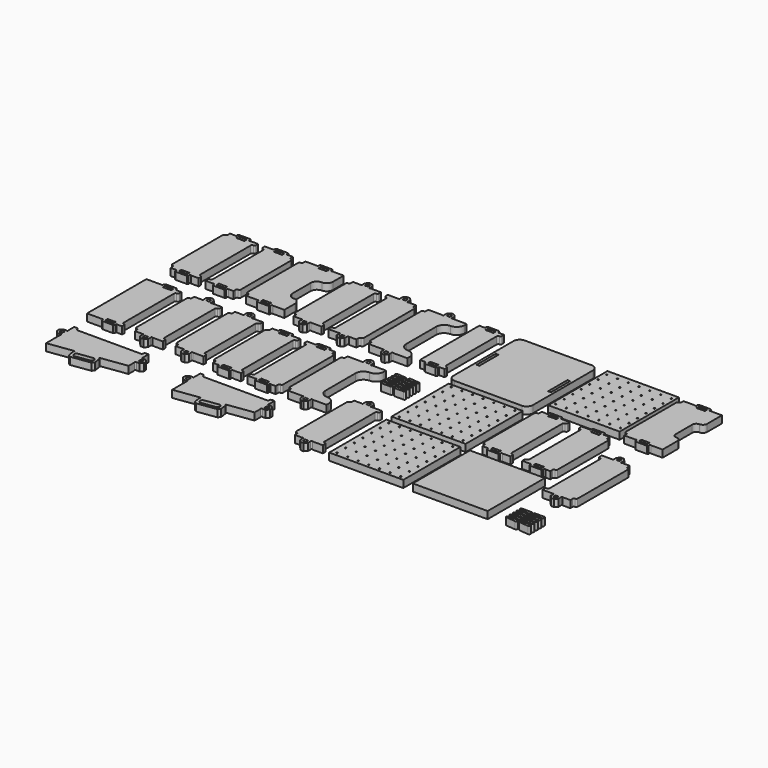
from build123d import *

# Parameters (mm, degrees)
F1_DEPTH = 35
F0_W     = 346.5
F0_H     = 359.2
F0_R     = 3.25
F0_W_2   = 363.004301
F0_H_2   = 346.5
F0_W_3   = 359.2


# Not quite as in the source:
# - ends of sketch curves that miss each other by under 0.0002 mm in the source are joined


with BuildPart() as f1:
    # F0 (on Top) → F1 (new body)
    with BuildSketch(Plane.XY):
        with BuildLine():
            Line((1149.792748, -503.188435), (1194.814221, -507.127303))
            ThreePointArc((1194.814221, -507.127303), (1198.6279509172, -505.8327167948), (1200.25, -502.14633))
            Line((1200.25, -502.14633), (1200.25, -497.715656))
            ThreePointArc((1200.25, -497.715656), (1198.7855339059, -494.1801220941), (1195.25, -492.715656))
            Line((1195.25, -492.715656), (1150.25, -492.715656))
            ThreePointArc((1150.25, -492.715656), (1145.0086213956, -497.7331831943), (1149.792748, -503.188435))
        make_face()
    extrude(amount=F1_DEPTH)


with BuildPart() as f1b:
    # F0 (on Top) → F1, piece 2 (new body)
    with BuildSketch(Plane.XY):
        with BuildLine():
            Line((1136.951296, -585.269026), (1136.951296, -580.838352))
            ThreePointArc((1136.951296, -580.838352), (1135.4868299059, -577.3028180941), (1131.951296, -575.838352))
            Line((1131.951296, -575.838352), (1086.951296, -575.838352))
            ThreePointArc((1086.951296, -575.838352), (1081.7099173757, -580.8558806483), (1086.4940449123, -586.3111320022))
            Line((1086.4940449123, -586.3111320022), (1131.515518, -590.25))
            ThreePointArc((1131.515518, -590.25), (1135.3292473166, -588.9554124289), (1136.951296, -585.269026))
        make_face()
    extrude(amount=F1_DEPTH)


with BuildPart() as f1c:
    # F0 (on Top) → F1, piece 3 (new body)
    with BuildSketch(Plane.XY):
        with BuildLine():
            Line((136.880955, -12.238569), (91.859482, -8.2997))
            ThreePointArc((91.859482, -8.2997), (88.0457520507, -9.5942872346), (86.423703, -13.280674))
            Line((86.423703, -13.280674), (86.423703, -17.711348))
            ThreePointArc((86.423703, -17.711348), (87.8881690941, -21.2468819059), (91.423703, -22.711348))
            Line((91.423703, -22.711348), (136.423703, -22.711348))
            ThreePointArc((136.423703, -22.711348), (141.6650816025, -17.6938198493), (136.880955, -12.238569))
        make_face()
    extrude(amount=F1_DEPTH)


with BuildPart() as f1d:
    # F0 (on Top) → F1, piece 4 (new body)
    with BuildSketch(Plane.XY):
        with BuildLine():
            ThreePointArc((23.125, -17.711348), (24.5894660941, -21.2468819059), (28.125, -22.711348))
            Line((28.125, -22.711348), (73.125, -22.711348))
            ThreePointArc((73.125, -22.711348), (78.3663786243, -17.6938193517), (73.5822510877, -12.2385679978))
            Line((73.5822510877, -12.2385679978), (28.560779, -8.2997))
            ThreePointArc((28.560779, -8.2997), (24.7470490507, -9.5942872346), (23.125, -13.280674))
            Line((23.125, -13.280674), (23.125, -17.711348))
        make_face()
    extrude(amount=F1_DEPTH)


with BuildPart() as f1e:
    # F0 (on Top) → F1, piece 5 (new body)
    with BuildSketch(Plane.XY):
        with BuildLine():
            ThreePointArc((73.125, -1.930674), (78.3663786243, 3.0868546483), (73.5822510877, 8.5421060022))
            Line((73.5822510877, 8.5421060022), (28.560779, 12.480974))
            ThreePointArc((28.560779, 12.480974), (24.7470490507, 11.1863867654), (23.125, 7.5))
            Line((23.125, 7.5), (23.125, 3.069326))
            ThreePointArc((23.125, 3.069326), (24.5894660941, -0.4662079059), (28.125, -1.930674))
            Line((28.125, -1.930674), (73.125, -1.930674))
        make_face()
    extrude(amount=F1_DEPTH)


with BuildPart() as f1f:
    # F0 (on Top) → F1, piece 6 (new body)
    with BuildSketch(Plane.XY):
        with BuildLine():
            Line((136.880955, 8.542105), (91.859482, 12.480974))
            ThreePointArc((91.859482, 12.480974), (88.0457520507, 11.1863867654), (86.423703, 7.5))
            Line((86.423703, 7.5), (86.423703, 3.069326))
            ThreePointArc((86.423703, 3.069326), (87.8881690941, -0.4662079059), (91.423703, -1.930674))
            Line((91.423703, -1.930674), (136.423703, -1.930674))
            ThreePointArc((136.423703, -1.930674), (141.6650816025, 3.0868541507), (136.880955, 8.542105))
        make_face()
    extrude(amount=F1_DEPTH)


with BuildPart() as f1g:
    # F0 (on Top) → F1, piece 7 (new body)
    with BuildSketch(Plane.XY):
        with BuildLine():
            Line((91.423703, 18.85), (136.423703, 18.85))
            ThreePointArc((136.423703, 18.85), (141.6650816025, 23.8675281507), (136.8809550801, 29.3227799154))
            Line((136.8809550801, 29.3227799154), (91.859482, 33.261648))
            ThreePointArc((91.859482, 33.261648), (88.0457520507, 31.9670607654), (86.423703, 28.280674))
            Line((86.423703, 28.280674), (86.423703, 23.85))
            ThreePointArc((86.423703, 23.85), (87.8881690941, 20.3144660941), (91.423703, 18.85))
        make_face()
    extrude(amount=F1_DEPTH)


with BuildPart() as f1h:
    # F0 (on Top) → F1, piece 8 (new body)
    with BuildSketch(Plane.XY):
        with BuildLine():
            Line((73.582251, 29.322779), (28.560779, 33.261648))
            ThreePointArc((28.560779, 33.261648), (24.7470490507, 31.9670607654), (23.125, 28.280674))
            Line((23.125, 28.280674), (23.125, 23.85))
            ThreePointArc((23.125, 23.85), (24.5894660941, 20.3144660941), (28.125, 18.85))
            Line((28.125, 18.85), (73.125, 18.85))
            ThreePointArc((73.125, 18.85), (78.3663786243, 23.8675286483), (73.582251, 29.322779))
        make_face()
    extrude(amount=F1_DEPTH)


with BuildPart() as f1i:
    # F0 (on Top) → F1, piece 9 (new body)
    with BuildSketch(Plane.XY):
        with BuildLine():
            Line((23.125, 49.061348), (23.125, 44.630674))
            ThreePointArc((23.125, 44.630674), (24.5894660941, 41.0951400941), (28.125, 39.630674))
            Line((28.125, 39.630674), (73.125, 39.630674))
            ThreePointArc((73.125, 39.630674), (78.3663786243, 44.6482026483), (73.5822510877, 50.1034540022))
            Line((73.5822510877, 50.1034540022), (28.560779, 54.042322))
            ThreePointArc((28.560779, 54.042322), (24.7470490507, 52.7477347654), (23.125, 49.061348))
        make_face()
    extrude(amount=F1_DEPTH)


with BuildPart() as f1j:
    # F0 (on Top) → F1, piece 10 (new body)
    with BuildSketch(Plane.XY):
        with BuildLine():
            ThreePointArc((86.423703, 44.630674), (87.8881690941, 41.0951400941), (91.423703, 39.630674))
            Line((91.423703, 39.630674), (136.423703, 39.630674))
            ThreePointArc((136.423703, 39.630674), (141.6650816025, 44.6482021507), (136.8809550801, 50.1034539154))
            Line((136.8809550801, 50.1034539154), (91.859482, 54.042322))
            ThreePointArc((91.859482, 54.042322), (88.0457520507, 52.7477347654), (86.423703, 49.061348))
            Line((86.423703, 49.061348), (86.423703, 44.630674))
        make_face()
    extrude(amount=F1_DEPTH)


with BuildPart() as f1k:
    # F0 (on Top) → F1, piece 11 (new body)
    with BuildSketch(Plane.XY):
        with BuildLine():
            Line((91.423703, 60.411348), (136.423703, 60.411348))
            ThreePointArc((136.423703, 60.411348), (141.6650816044, 65.4288761943), (136.8809549933, 70.8841279229))
            Line((136.8809549933, 70.8841279229), (91.859482, 74.822996))
            ThreePointArc((91.859482, 74.822996), (88.0457520828, 73.5284097948), (86.423703, 69.842023))
            Line((86.423703, 69.842023), (86.423703, 65.411348))
            ThreePointArc((86.423703, 65.411348), (87.8881690941, 61.8758140941), (91.423703, 60.411348))
        make_face()
    extrude(amount=F1_DEPTH)


with BuildPart() as f1l:
    # F0 (on Top) → F1, piece 12 (new body)
    with BuildSketch(Plane.XY):
        with BuildLine():
            Line((73.582251, 70.884128), (28.560779, 74.822996))
            ThreePointArc((28.560779, 74.822996), (24.7470490828, 73.5284097948), (23.125, 69.842023))
            Line((23.125, 69.842023), (23.125, 65.411348))
            ThreePointArc((23.125, 65.411348), (24.5894660941, 61.8758140941), (28.125, 60.411348))
            Line((28.125, 60.411348), (73.125, 60.411348))
            ThreePointArc((73.125, 60.411348), (78.3663786262, 65.4288766919), (73.582251, 70.884128))
        make_face()
    extrude(amount=F1_DEPTH)


with BuildPart() as f1m:
    # F0 (on Top) → F1, piece 13 (new body)
    with BuildSketch(Plane.XY):
        with BuildLine():
            Line((1149.792748, -523.969109), (1194.814221, -527.907977))
            ThreePointArc((1194.814221, -527.907977), (1198.6279509172, -526.6133907948), (1200.25, -522.927004))
            Line((1200.25, -522.927004), (1200.25, -518.49633))
            ThreePointArc((1200.25, -518.49633), (1198.7855339059, -514.9607960941), (1195.25, -513.49633))
            Line((1195.25, -513.49633), (1150.25, -513.49633))
            ThreePointArc((1150.25, -513.49633), (1145.0086213956, -518.5138571943), (1149.792748, -523.969109))
        make_face()
    extrude(amount=F1_DEPTH)


with BuildPart() as f1n:
    # F0 (on Top) → F1, piece 14 (new body)
    with BuildSketch(Plane.XY):
        with BuildLine():
            Line((1195.25, -534.277004), (1150.25, -534.277004))
            ThreePointArc((1150.25, -534.277004), (1145.0086213975, -539.2945321507), (1149.7927479199, -544.7497839154))
            Line((1149.7927479199, -544.7497839154), (1194.814221, -548.688652))
            ThreePointArc((1194.814221, -548.688652), (1198.6279509493, -547.3940647654), (1200.25, -543.707678))
            Line((1200.25, -543.707678), (1200.25, -539.277004))
            ThreePointArc((1200.25, -539.277004), (1198.7855339059, -535.7414700941), (1195.25, -534.277004))
        make_face()
    extrude(amount=F1_DEPTH)


with BuildPart() as f1o:
    # F0 (on Top) → F1, piece 15 (new body)
    with BuildSketch(Plane.XY):
        with BuildLine():
            Line((1149.792748, -565.530457), (1194.814221, -569.469326))
            ThreePointArc((1194.814221, -569.469326), (1198.6279509493, -568.1747387654), (1200.25, -564.488352))
            Line((1200.25, -564.488352), (1200.25, -560.057678))
            ThreePointArc((1200.25, -560.057678), (1198.7855339059, -556.5221440941), (1195.25, -555.057678))
            Line((1195.25, -555.057678), (1150.25, -555.057678))
            ThreePointArc((1150.25, -555.057678), (1145.0086213975, -560.0752061507), (1149.792748, -565.530457))
        make_face()
    extrude(amount=F1_DEPTH)


with BuildPart() as f1p:
    # F0 (on Top) → F1, piece 16 (new body)
    with BuildSketch(Plane.XY):
        with BuildLine():
            Line((1195.25, -575.838352), (1150.25, -575.838352))
            ThreePointArc((1150.25, -575.838352), (1145.0086213975, -580.8558801507), (1149.7927479199, -586.3111319154))
            Line((1149.7927479199, -586.3111319154), (1194.814221, -590.25))
            ThreePointArc((1194.814221, -590.25), (1198.6279509493, -588.9554127654), (1200.25, -585.269026))
            Line((1200.25, -585.269026), (1200.25, -580.838352))
            ThreePointArc((1200.25, -580.838352), (1198.7855339059, -577.3028180941), (1195.25, -575.838352))
        make_face()
    extrude(amount=F1_DEPTH)


with BuildPart() as f1q:
    # F0 (on Top) → F1, piece 17 (new body)
    with BuildSketch(Plane.XY):
        with BuildLine():
            Line((1086.494045, -565.530457), (1131.515518, -569.469326))
            ThreePointArc((1131.515518, -569.469326), (1135.3292473166, -568.1747384289), (1136.951296, -564.488352))
            Line((1136.951296, -564.488352), (1136.951296, -560.057678))
            ThreePointArc((1136.951296, -560.057678), (1135.4868299059, -556.5221440941), (1131.951296, -555.057678))
            Line((1131.951296, -555.057678), (1086.951296, -555.057678))
            ThreePointArc((1086.951296, -555.057678), (1081.7099173757, -560.0752066483), (1086.494045, -565.530457))
        make_face()
    extrude(amount=F1_DEPTH)


with BuildPart() as f1r:
    # F0 (on Top) → F1, piece 18 (new body)
    with BuildSketch(Plane.XY):
        with BuildLine():
            Line((1086.494045, -544.749783), (1131.515518, -548.688652))
            ThreePointArc((1131.515518, -548.688652), (1135.3292473166, -547.3940644289), (1136.951296, -543.707678))
            Line((1136.951296, -543.707678), (1136.951296, -539.277004))
            ThreePointArc((1136.951296, -539.277004), (1135.4868299059, -535.7414700941), (1131.951296, -534.277004))
            Line((1131.951296, -534.277004), (1086.951296, -534.277004))
            ThreePointArc((1086.951296, -534.277004), (1081.7099173757, -539.2945326483), (1086.494045, -544.749783))
        make_face()
    extrude(amount=F1_DEPTH)


with BuildPart() as f1s:
    # F0 (on Top) → F1, piece 19 (new body)
    with BuildSketch(Plane.XY):
        with BuildLine():
            Line((1086.494045, -523.969109), (1131.515518, -527.907977))
            ThreePointArc((1131.515518, -527.907977), (1135.3292472844, -526.6133904583), (1136.951296, -522.927004))
            Line((1136.951296, -522.927004), (1136.951296, -518.49633))
            ThreePointArc((1136.951296, -518.49633), (1135.4868299059, -514.9607960941), (1131.951296, -513.49633))
            Line((1131.951296, -513.49633), (1086.951296, -513.49633))
            ThreePointArc((1086.951296, -513.49633), (1081.7099173738, -518.5138576919), (1086.494045, -523.969109))
        make_face()
    extrude(amount=F1_DEPTH)


with BuildPart() as f1t:
    # F0 (on Top) → F1, piece 20 (new body)
    with BuildSketch(Plane.XY):
        with BuildLine():
            ThreePointArc((1136.951296, -497.715656), (1135.4868299059, -494.1801220941), (1131.951296, -492.715656))
            Line((1131.951296, -492.715656), (1086.951296, -492.715656))
            ThreePointArc((1086.951296, -492.715656), (1081.7099173738, -497.7331836919), (1086.4940449991, -503.1884350098))
            Line((1086.4940449991, -503.1884350098), (1131.515518, -507.127303))
            ThreePointArc((1131.515518, -507.127303), (1135.3292472844, -505.8327164583), (1136.951296, -502.14633))
            Line((1136.951296, -502.14633), (1136.951296, -497.715656))
        make_face()
    extrude(amount=F1_DEPTH)


with BuildPart() as f1u:
    # F0 (on Top) → F1, piece 21 (new body)
    with BuildSketch(Plane.XY):
        with Locations((808.0625, 410.65)):
            Rectangle(F0_W, F0_H)
        with Locations((650.8325, 256.07)):
            Circle(F0_R, mode=Mode.SUBTRACT)
        with Locations((703.2425, 256.07)):
            Circle(F0_R, mode=Mode.SUBTRACT)
        with Locations((755.6525, 256.07)):
            Circle(F0_R, mode=Mode.SUBTRACT)
        with Locations((808.0625, 256.07)):
            Circle(F0_R, mode=Mode.SUBTRACT)
        with Locations((860.4725, 256.07)):
            Circle(F0_R, mode=Mode.SUBTRACT)
        with Locations((912.8825, 256.07)):
            Circle(F0_R, mode=Mode.SUBTRACT)
        with Locations((965.2925, 256.07)):
            Circle(F0_R, mode=Mode.SUBTRACT)
        with Locations((650.8325, 307.596667)):
            Circle(F0_R, mode=Mode.SUBTRACT)
        with Locations((703.2425, 307.596667)):
            Circle(F0_R, mode=Mode.SUBTRACT)
        with Locations((650.8325, 359.123334)):
            Circle(F0_R, mode=Mode.SUBTRACT)
        with Locations((703.2425, 359.123334)):
            Circle(F0_R, mode=Mode.SUBTRACT)
        with Locations((755.6525, 307.596667)):
            Circle(F0_R, mode=Mode.SUBTRACT)
        with Locations((808.0625, 307.596667)):
            Circle(F0_R, mode=Mode.SUBTRACT)
        with Locations((860.4725, 307.596667)):
            Circle(F0_R, mode=Mode.SUBTRACT)
        with Locations((755.6525, 359.123334)):
            Circle(F0_R, mode=Mode.SUBTRACT)
        with Locations((808.0625, 359.123334)):
            Circle(F0_R, mode=Mode.SUBTRACT)
        with Locations((860.4725, 359.123334)):
            Circle(F0_R, mode=Mode.SUBTRACT)
        with Locations((650.8325, 410.65)):
            Circle(F0_R, mode=Mode.SUBTRACT)
        with Locations((703.2425, 410.65)):
            Circle(F0_R, mode=Mode.SUBTRACT)
        with Locations((755.6525, 410.65)):
            Circle(F0_R, mode=Mode.SUBTRACT)
        with Locations((808.0625, 410.65)):
            Circle(F0_R, mode=Mode.SUBTRACT)
        with Locations((860.4725, 410.65)):
            Circle(F0_R, mode=Mode.SUBTRACT)
        with Locations((912.8825, 307.596667)):
            Circle(F0_R, mode=Mode.SUBTRACT)
        with Locations((965.2925, 307.596667)):
            Circle(F0_R, mode=Mode.SUBTRACT)
        with Locations((912.8825, 359.123334)):
            Circle(F0_R, mode=Mode.SUBTRACT)
        with Locations((965.2925, 359.123334)):
            Circle(F0_R, mode=Mode.SUBTRACT)
        with Locations((912.8825, 410.65)):
            Circle(F0_R, mode=Mode.SUBTRACT)
        with Locations((965.2925, 410.65)):
            Circle(F0_R, mode=Mode.SUBTRACT)
        with Locations((650.8325, 462.176667)):
            Circle(F0_R, mode=Mode.SUBTRACT)
        with Locations((703.2425, 462.176667)):
            Circle(F0_R, mode=Mode.SUBTRACT)
        with Locations((650.8325, 513.703334)):
            Circle(F0_R, mode=Mode.SUBTRACT)
        with Locations((703.2425, 513.703334)):
            Circle(F0_R, mode=Mode.SUBTRACT)
        with Locations((755.6525, 462.176667)):
            Circle(F0_R, mode=Mode.SUBTRACT)
        with Locations((808.0625, 462.176667)):
            Circle(F0_R, mode=Mode.SUBTRACT)
        with Locations((860.4725, 462.176667)):
            Circle(F0_R, mode=Mode.SUBTRACT)
        with Locations((755.6525, 513.703334)):
            Circle(F0_R, mode=Mode.SUBTRACT)
        with Locations((808.0625, 513.703334)):
            Circle(F0_R, mode=Mode.SUBTRACT)
        with Locations((860.4725, 513.703334)):
            Circle(F0_R, mode=Mode.SUBTRACT)
        with Locations((650.8325, 565.23)):
            Circle(F0_R, mode=Mode.SUBTRACT)
        with Locations((703.2425, 565.23)):
            Circle(F0_R, mode=Mode.SUBTRACT)
        with Locations((755.6525, 565.23)):
            Circle(F0_R, mode=Mode.SUBTRACT)
        with Locations((808.0625, 565.23)):
            Circle(F0_R, mode=Mode.SUBTRACT)
        with Locations((860.4725, 565.23)):
            Circle(F0_R, mode=Mode.SUBTRACT)
        with Locations((912.8825, 462.176667)):
            Circle(F0_R, mode=Mode.SUBTRACT)
        with Locations((965.2925, 462.176667)):
            Circle(F0_R, mode=Mode.SUBTRACT)
        with Locations((912.8825, 513.703334)):
            Circle(F0_R, mode=Mode.SUBTRACT)
        with Locations((965.2925, 513.703334)):
            Circle(F0_R, mode=Mode.SUBTRACT)
        with Locations((912.8825, 565.23)):
            Circle(F0_R, mode=Mode.SUBTRACT)
        with Locations((965.2925, 565.23)):
            Circle(F0_R, mode=Mode.SUBTRACT)
    extrude(amount=F1_DEPTH)


with BuildPart() as f1v:
    # F0 (on Top) → F1, piece 22 (new body)
    with BuildSketch(Plane.XY):
        with BuildLine():
            Line((1014.25, 577.55), (1014.25, 564.45))
            ThreePointArc((1014.25, 564.45), (1012.1997474683, 559.5002525317), (1007.25, 557.45))
            ThreePointArc((1007.25, 557.45), (1002.3002525317, 555.3997474683), (1000.25, 550.45))
            Line((1000.25, 550.45), (1000.25, 244.65))
            ThreePointArc((1000.25, 244.65), (1002.3002525317, 239.7002525317), (1007.25, 237.65))
            ThreePointArc((1007.25, 237.65), (1012.1997474683, 235.5997474683), (1014.25, 230.65))
            Line((1014.25, 230.65), (1014.25, 217.55))
            Line((1014.25, 217.55), (1070.046279, 217.55))
            ThreePointArc((1070.046279, 217.55), (1070.3820500038, 217.6080563536), (1070.6788337273, 217.7754843339))
            ThreePointArc((1070.6788337273, 217.7754843339), (1075.1600001831, 217.5500001831), (1075.3854841076, 213.0688339121))
            ThreePointArc((1075.3854841076, 213.0688339121), (1075.2180562235, 212.772050639), (1075.16, 212.43628))
            Line((1075.16, 212.43628), (1075.16, 208.64314))
            Line((1075.16, 208.64314), (1078.95314, 204.85))
            Line((1078.95314, 204.85), (1135.54686, 204.85))
            Line((1135.54686, 204.85), (1139.34, 208.64314))
            Line((1139.34, 208.64314), (1139.34, 212.43628))
            ThreePointArc((1139.34, 212.43628), (1139.2819437765, 212.772050639), (1139.114516156, 213.0688341274))
            ThreePointArc((1139.114516156, 213.0688341274), (1139.3399998169, 217.5500001831), (1143.8211660879, 217.7754841076))
            ThreePointArc((1143.8211660879, 217.7754841076), (1144.117949361, 217.6080562235), (1144.45372, 217.55))
            Line((1144.45372, 217.55), (1200.25, 217.55))
            Line((1200.25, 217.55), (1200.25, 307.55))
            ThreePointArc((1200.25, 307.55), (1194.3921356237, 321.6921356237), (1180.25, 327.55))
            ThreePointArc((1180.25, 327.55), (1166.1078643763, 333.4078643763), (1160.25, 347.55))
            Line((1160.25, 347.55), (1160.25, 447.55))
            ThreePointArc((1160.25, 447.55), (1166.1078643763, 461.6921356237), (1180.25, 467.55))
            ThreePointArc((1180.25, 467.55), (1194.3921356237, 473.4078643763), (1200.25, 487.55))
            Line((1200.25, 487.55), (1200.25, 577.55))
            Line((1200.25, 577.55), (1144.45372, 577.55))
            ThreePointArc((1144.45372, 577.55), (1144.117949361, 577.4919437765), (1143.8211658726, 577.324516156))
            ThreePointArc((1143.8211658726, 577.324516156), (1139.3399998169, 577.5499998169), (1139.1145158924, 582.0311660879))
            ThreePointArc((1139.1145158924, 582.0311660879), (1139.2819436464, 582.3279499962), (1139.34, 582.663721))
            Line((1139.34, 582.663721), (1139.34, 586.456861))
            Line((1139.34, 586.456861), (1135.54686, 590.25))
            Line((1135.54686, 590.25), (1078.95314, 590.25))
            Line((1078.95314, 590.25), (1075.16, 586.456861))
            Line((1075.16, 586.456861), (1075.16, 582.663721))
            ThreePointArc((1075.16, 582.663721), (1075.2180563536, 582.3279499962), (1075.3854843339, 582.0311662727))
            ThreePointArc((1075.3854843339, 582.0311662727), (1075.1600001831, 577.5499998169), (1070.6788339121, 577.3245158924))
            ThreePointArc((1070.6788339121, 577.3245158924), (1070.3820500038, 577.4919436464), (1070.046279, 577.55))
            Line((1070.046279, 577.55), (1014.25, 577.55))
        make_face()
        with BuildLine():
            Line((1121.526279, 217.38), (1092.97372, 217.38))
            ThreePointArc((1092.97372, 217.38), (1092.637949361, 217.3219437765), (1092.3411658726, 217.154516156))
            ThreePointArc((1092.3411658726, 217.154516156), (1087.8599998169, 217.3799998169), (1087.6345158924, 221.8611660879))
            ThreePointArc((1087.6345158924, 221.8611660879), (1087.8019436464, 222.1579499962), (1087.86, 222.493721))
            Line((1087.86, 222.493721), (1087.86, 225.30628))
            ThreePointArc((1087.86, 225.30628), (1087.8019437765, 225.642050639), (1087.634516156, 225.9388341274))
            ThreePointArc((1087.634516156, 225.9388341274), (1087.8599998169, 230.4200001831), (1092.3411660879, 230.6454841076))
            ThreePointArc((1092.3411660879, 230.6454841076), (1092.637949361, 230.4780562235), (1092.97372, 230.42))
            Line((1092.97372, 230.42), (1121.526279, 230.42))
            ThreePointArc((1121.526279, 230.42), (1121.8620500038, 230.4780563536), (1122.1588337273, 230.6454843339))
            ThreePointArc((1122.1588337273, 230.6454843339), (1126.6400001831, 230.4200001831), (1126.8654841076, 225.9388339121))
            ThreePointArc((1126.8654841076, 225.9388339121), (1126.6980562235, 225.642050639), (1126.64, 225.30628))
            Line((1126.64, 225.30628), (1126.64, 222.493721))
            ThreePointArc((1126.64, 222.493721), (1126.6980563536, 222.1579499962), (1126.8654843339, 221.8611662727))
            ThreePointArc((1126.8654843339, 221.8611662727), (1126.6400001831, 217.3799998169), (1122.1588339121, 217.1545158924))
            ThreePointArc((1122.1588339121, 217.1545158924), (1121.8620500038, 217.3219436464), (1121.526279, 217.38))
        make_face(mode=Mode.SUBTRACT)
        with BuildLine():
            Line((1087.86, 569.793721), (1087.86, 572.60628))
            ThreePointArc((1087.86, 572.60628), (1087.8019437765, 572.942050639), (1087.634516156, 573.2388341274))
            ThreePointArc((1087.634516156, 573.2388341274), (1087.8599998169, 577.7200001831), (1092.3411660879, 577.9454841076))
            ThreePointArc((1092.3411660879, 577.9454841076), (1092.637949361, 577.7780562235), (1092.97372, 577.72))
            Line((1092.97372, 577.72), (1121.526279, 577.72))
            ThreePointArc((1121.526279, 577.72), (1121.8620500038, 577.7780563536), (1122.1588337273, 577.9454843339))
            ThreePointArc((1122.1588337273, 577.9454843339), (1126.6400001831, 577.7200001831), (1126.8654841076, 573.2388339121))
            ThreePointArc((1126.8654841076, 573.2388339121), (1126.6980562235, 572.942050639), (1126.64, 572.60628))
            Line((1126.64, 572.60628), (1126.64, 569.793721))
            ThreePointArc((1126.64, 569.793721), (1126.6980563536, 569.4579499962), (1126.8654843339, 569.1611662727))
            ThreePointArc((1126.8654843339, 569.1611662727), (1126.6400001831, 564.6799998169), (1122.1588339121, 564.4545158924))
            ThreePointArc((1122.1588339121, 564.4545158924), (1121.8620500038, 564.6219436464), (1121.526279, 564.68))
            Line((1121.526279, 564.68), (1092.97372, 564.68))
            ThreePointArc((1092.97372, 564.68), (1092.637949361, 564.6219437765), (1092.3411658726, 564.454516156))
            ThreePointArc((1092.3411658726, 564.454516156), (1087.8599998169, 564.6799998169), (1087.6345158924, 569.1611660879))
            ThreePointArc((1087.6345158924, 569.1611660879), (1087.8019436464, 569.4579499962), (1087.86, 569.793721))
        make_face(mode=Mode.SUBTRACT)
    extrude(amount=F1_DEPTH)


with BuildPart() as f1w:
    # F0 (on Top) → F1, piece 23 (new body)
    with BuildSketch(Plane.XY):
        with BuildLine():
            ThreePointArc((1144.3653558834, -328.5538791065), (1144.4699998169, -323.9328278169), (1149.0910511065, -323.8281838834))
            ThreePointArc((1149.0910511065, -323.8281838834), (1149.2161329582, -323.9057504553), (1149.360801, -323.932828))
            Line((1149.360801, -323.932828), (1186.25, -323.932828))
            Line((1186.25, -323.932828), (1186.25, -310.832828))
            ThreePointArc((1186.25, -310.832828), (1188.3002525317, -305.8830805317), (1193.25, -303.832828))
            ThreePointArc((1193.25, -303.832828), (1198.1997474683, -301.7825754683), (1200.25, -296.832828))
            Line((1200.25, -296.832828), (1200.25, 8.967172))
            ThreePointArc((1200.25, 8.967172), (1198.1997474683, 13.9169194683), (1193.25, 15.967172))
            ThreePointArc((1193.25, 15.967172), (1188.3002525317, 18.0174245317), (1186.25, 22.967172))
            Line((1186.25, 22.967172), (1186.25, 36.067172))
            Line((1186.25, 36.067172), (1149.360801, 36.067172))
            ThreePointArc((1149.360801, 36.067172), (1149.2161329582, 36.0400944553), (1149.0910511932, 35.9625277884))
            ThreePointArc((1149.0910511932, 35.9625277884), (1144.4699995559, 36.067172078), (1144.3653563814, 40.6882236517))
            ThreePointArc((1144.3653563814, 40.6882236517), (1144.4429225888, 40.8133053024), (1144.47, 40.957973))
            Line((1144.47, 40.957973), (1144.47, 55.376371))
            Line((1144.47, 55.376371), (1132.229199, 67.617172))
            Line((1132.229199, 67.617172), (1118.270801, 67.617172))
            Line((1118.270801, 67.617172), (1106.03, 55.376371))
            Line((1106.03, 55.376371), (1106.03, 40.957973))
            ThreePointArc((1106.03, 40.957973), (1106.0570774112, 40.8133053024), (1106.1346437136, 40.6882237385))
            ThreePointArc((1106.1346437136, 40.6882237385), (1106.0300001831, 36.0671718169), (1101.4089483483, 35.9625283814))
            ThreePointArc((1101.4089483483, 35.9625283814), (1101.2838666976, 36.0400945888), (1101.139199, 36.067172))
            Line((1101.139199, 36.067172), (1050.25, 36.067172))
            Line((1050.25, 36.067172), (1050.25, 23.367172))
            ThreePointArc((1050.25, 23.367172), (1052.3002525317, 18.4174245317), (1057.25, 16.367172))
            ThreePointArc((1057.25, 16.367172), (1062.1997474683, 14.3169194683), (1064.25, 9.367172))
            Line((1064.25, 9.367172), (1064.25, -297.232828))
            ThreePointArc((1064.25, -297.232828), (1062.1997474683, -302.1825754683), (1057.25, -304.232828))
            ThreePointArc((1057.25, -304.232828), (1052.3002525317, -306.2830805317), (1050.25, -311.232828))
            Line((1050.25, -311.232828), (1050.25, -323.932828))
            Line((1050.25, -323.932828), (1101.139199, -323.932828))
            ThreePointArc((1101.139199, -323.932828), (1101.2838666976, -323.9057505888), (1101.4089482615, -323.8281842864))
            ThreePointArc((1101.4089482615, -323.8281842864), (1106.029999922, -323.9328275559), (1106.1346441166, -328.5538791065))
            ThreePointArc((1106.1346441166, -328.5538791065), (1106.0570775447, -328.6789609582), (1106.03, -328.823629))
            Line((1106.03, -328.823629), (1106.03, -343.242027))
            Line((1106.03, -343.242027), (1118.270801, -355.482828))
            Line((1118.270801, -355.482828), (1132.229199, -355.482828))
            Line((1132.229199, -355.482828), (1144.47, -343.242027))
            Line((1144.47, -343.242027), (1144.47, -328.823629))
            ThreePointArc((1144.47, -328.823629), (1144.4429224553, -328.6789609582), (1144.3653558834, -328.5538791065))
        make_face()
        with BuildLine():
            Line((1131.77, -334.173629), (1131.77, -337.892027))
            ThreePointArc((1131.77, -337.892027), (1131.7970774112, -338.0366946976), (1131.8746437136, -338.1617762615))
            ThreePointArc((1131.8746437136, -338.1617762615), (1131.7700001831, -342.7828281831), (1127.1489483483, -342.8874716186))
            ThreePointArc((1127.1489483483, -342.8874716186), (1127.0238666976, -342.8099054112), (1126.879199, -342.782828))
            Line((1126.879199, -342.782828), (1123.620801, -342.782828))
            ThreePointArc((1123.620801, -342.782828), (1123.4761329582, -342.8099055447), (1123.3510511932, -342.8874722116))
            ThreePointArc((1123.3510511932, -342.8874722116), (1118.7299995559, -342.782827922), (1118.6253563814, -338.1617763483))
            ThreePointArc((1118.6253563814, -338.1617763483), (1118.7029225888, -338.0366946976), (1118.73, -337.892027))
            Line((1118.73, -337.892027), (1118.73, -334.173629))
            ThreePointArc((1118.73, -334.173629), (1118.7029224553, -334.0289609582), (1118.6253557884, -333.9038791932))
            ThreePointArc((1118.6253557884, -333.9038791932), (1118.7299998169, -329.2828278169), (1123.3510511065, -329.1781838834))
            ThreePointArc((1123.3510511065, -329.1781838834), (1123.4761329582, -329.2557504553), (1123.620801, -329.282828))
            Line((1123.620801, -329.282828), (1126.879199, -329.282828))
            ThreePointArc((1126.879199, -329.282828), (1127.0238666976, -329.2557505888), (1127.1489482615, -329.1781842864))
            ThreePointArc((1127.1489482615, -329.1781842864), (1131.769999922, -329.2828275559), (1131.8746441166, -333.9038791065))
            ThreePointArc((1131.8746441166, -333.9038791065), (1131.7970775447, -334.0289609582), (1131.77, -334.173629))
        make_face(mode=Mode.SUBTRACT)
        with BuildLine():
            ThreePointArc((1118.6253558834, 50.2961208935), (1118.7299998169, 54.9171721831), (1123.3510511065, 55.0218161166))
            ThreePointArc((1123.3510511065, 55.0218161166), (1123.4761329582, 54.9442495447), (1123.620801, 54.917172))
            Line((1123.620801, 54.917172), (1126.879199, 54.917172))
            ThreePointArc((1126.879199, 54.917172), (1127.0238666976, 54.9442494112), (1127.1489482615, 55.0218157136))
            ThreePointArc((1127.1489482615, 55.0218157136), (1131.769999922, 54.9171724441), (1131.8746441166, 50.2961208935))
            ThreePointArc((1131.8746441166, 50.2961208935), (1131.7970775447, 50.1710390418), (1131.77, 50.026371))
            Line((1131.77, 50.026371), (1131.77, 46.307973))
            ThreePointArc((1131.77, 46.307973), (1131.7970774112, 46.1633053024), (1131.8746437136, 46.0382237385))
            ThreePointArc((1131.8746437136, 46.0382237385), (1131.7700001831, 41.4171718169), (1127.1489483483, 41.3125283814))
            ThreePointArc((1127.1489483483, 41.3125283814), (1127.0238666976, 41.3900945888), (1126.879199, 41.417172))
            Line((1126.879199, 41.417172), (1123.620801, 41.417172))
            ThreePointArc((1123.620801, 41.417172), (1123.4761329582, 41.3900944553), (1123.3510511932, 41.3125277884))
            ThreePointArc((1123.3510511932, 41.3125277884), (1118.7299995559, 41.417172078), (1118.6253563814, 46.0382236517))
            ThreePointArc((1118.6253563814, 46.0382236517), (1118.7029225888, 46.1633053024), (1118.73, 46.307973))
            Line((1118.73, 46.307973), (1118.73, 50.026371))
            ThreePointArc((1118.73, 50.026371), (1118.7029224553, 50.1710390418), (1118.6253558834, 50.2961208935))
        make_face(mode=Mode.SUBTRACT)
    extrude(amount=F1_DEPTH)


with BuildPart() as f1x:
    # F0 (on Top) → F1, piece 24 (new body)
    with BuildSketch(Plane.XY):
        with BuildLine():
            Line((978.53125, -186.35), (978.53125, -173.25))
            ThreePointArc((978.53125, -173.25), (980.5815025317, -168.3002525317), (985.53125, -166.25))
            ThreePointArc((985.53125, -166.25), (990.4809974683, -164.1997474683), (992.53125, -159.25))
            Line((992.53125, -159.25), (992.53125, 146.55))
            ThreePointArc((992.53125, 146.55), (990.4809974683, 151.4997474683), (985.53125, 153.55))
            ThreePointArc((985.53125, 153.55), (980.5815025317, 155.6002525317), (978.53125, 160.55))
            Line((978.53125, 160.55), (978.53125, 173.65))
            Line((978.53125, 173.65), (954.73497, 173.65))
            ThreePointArc((954.73497, 173.65), (954.399199361, 173.5919437765), (954.1024158726, 173.424516156))
            ThreePointArc((954.1024158726, 173.424516156), (949.6212498169, 173.6499998169), (949.3957658924, 178.1311660879))
            ThreePointArc((949.3957658924, 178.1311660879), (949.5631936464, 178.4279499962), (949.62125, 178.763721))
            Line((949.62125, 178.763721), (949.62125, 182.556861))
            Line((949.62125, 182.556861), (945.82811, 186.35))
            Line((945.82811, 186.35), (889.23439, 186.35))
            Line((889.23439, 186.35), (885.44125, 182.556861))
            Line((885.44125, 182.556861), (885.44125, 178.763721))
            ThreePointArc((885.44125, 178.763721), (885.4993063536, 178.4279499962), (885.6667343339, 178.1311662727))
            ThreePointArc((885.6667343339, 178.1311662727), (885.4412501831, 173.6499998169), (880.9600839121, 173.4245158924))
            ThreePointArc((880.9600839121, 173.4245158924), (880.6633000038, 173.5919436464), (880.327529, 173.65))
            Line((880.327529, 173.65), (842.53125, 173.65))
            Line((842.53125, 173.65), (842.53125, 160.95))
            ThreePointArc((842.53125, 160.95), (844.5815025317, 156.0002525317), (849.53125, 153.95))
            ThreePointArc((849.53125, 153.95), (854.4809974683, 151.8997474683), (856.53125, 146.95))
            Line((856.53125, 146.95), (856.53125, -159.65))
            ThreePointArc((856.53125, -159.65), (854.4809974683, -164.5997474683), (849.53125, -166.65))
            ThreePointArc((849.53125, -166.65), (844.5815025317, -168.7002525317), (842.53125, -173.65))
            Line((842.53125, -173.65), (842.53125, -186.35))
            Line((842.53125, -186.35), (880.327529, -186.35))
            ThreePointArc((880.327529, -186.35), (880.6633000038, -186.2919436464), (880.9600837273, -186.1245156661))
            ThreePointArc((880.9600837273, -186.1245156661), (885.4412501831, -186.3499998169), (885.6667341076, -190.8311660879))
            ThreePointArc((885.6667341076, -190.8311660879), (885.4993062235, -191.127949361), (885.44125, -191.46372))
            Line((885.44125, -191.46372), (885.44125, -195.25686))
            Line((885.44125, -195.25686), (889.23439, -199.05))
            Line((889.23439, -199.05), (945.82811, -199.05))
            Line((945.82811, -199.05), (949.62125, -195.25686))
            Line((949.62125, -195.25686), (949.62125, -191.46372))
            ThreePointArc((949.62125, -191.46372), (949.5631937765, -191.127949361), (949.395766156, -190.8311658726))
            ThreePointArc((949.395766156, -190.8311658726), (949.6212498169, -186.3499998169), (954.1024160879, -186.1245158924))
            ThreePointArc((954.1024160879, -186.1245158924), (954.399199361, -186.2919437765), (954.73497, -186.35))
            Line((954.73497, -186.35), (978.53125, -186.35))
        make_face()
        with BuildLine():
            Line((936.92125, -178.59372), (936.92125, -181.406279))
            ThreePointArc((936.92125, -181.406279), (936.9793063536, -181.7420500038), (937.1467343339, -182.0388337273))
            ThreePointArc((937.1467343339, -182.0388337273), (936.9212501831, -186.5200001831), (932.4400839121, -186.7454841076))
            ThreePointArc((932.4400839121, -186.7454841076), (932.1433000038, -186.5780563536), (931.807529, -186.52))
            Line((931.807529, -186.52), (903.25497, -186.52))
            ThreePointArc((903.25497, -186.52), (902.919199361, -186.5780562235), (902.6224158726, -186.745483844))
            ThreePointArc((902.6224158726, -186.745483844), (898.1412498169, -186.5200001831), (897.9157658924, -182.0388339121))
            ThreePointArc((897.9157658924, -182.0388339121), (898.0831936464, -181.7420500038), (898.14125, -181.406279))
            Line((898.14125, -181.406279), (898.14125, -178.59372))
            ThreePointArc((898.14125, -178.59372), (898.0831937765, -178.257949361), (897.915766156, -177.9611658726))
            ThreePointArc((897.915766156, -177.9611658726), (898.1412498169, -173.4799998169), (902.6224160879, -173.2545158924))
            ThreePointArc((902.6224160879, -173.2545158924), (902.919199361, -173.4219437765), (903.25497, -173.48))
            Line((903.25497, -173.48), (931.807529, -173.48))
            ThreePointArc((931.807529, -173.48), (932.1433000038, -173.4219436464), (932.4400837273, -173.2545156661))
            ThreePointArc((932.4400837273, -173.2545156661), (936.9212501831, -173.4799998169), (937.1467341076, -177.9611660879))
            ThreePointArc((937.1467341076, -177.9611660879), (936.9793062235, -178.257949361), (936.92125, -178.59372))
        make_face(mode=Mode.SUBTRACT)
        with BuildLine():
            Line((903.25497, 173.82), (931.807529, 173.82))
            ThreePointArc((931.807529, 173.82), (932.1433000038, 173.8780563536), (932.4400837273, 174.0454843339))
            ThreePointArc((932.4400837273, 174.0454843339), (936.9212501831, 173.8200001831), (937.1467341076, 169.3388339121))
            ThreePointArc((937.1467341076, 169.3388339121), (936.9793062235, 169.042050639), (936.92125, 168.70628))
            Line((936.92125, 168.70628), (936.92125, 165.893721))
            ThreePointArc((936.92125, 165.893721), (936.9793063536, 165.5579499962), (937.1467343339, 165.2611662727))
            ThreePointArc((937.1467343339, 165.2611662727), (936.9212501831, 160.7799998169), (932.4400839121, 160.5545158924))
            ThreePointArc((932.4400839121, 160.5545158924), (932.1433000038, 160.7219436464), (931.807529, 160.78))
            Line((931.807529, 160.78), (903.25497, 160.78))
            ThreePointArc((903.25497, 160.78), (902.919199361, 160.7219437765), (902.6224158726, 160.554516156))
            ThreePointArc((902.6224158726, 160.554516156), (898.1412498169, 160.7799998169), (897.9157658924, 165.2611660879))
            ThreePointArc((897.9157658924, 165.2611660879), (898.0831936464, 165.5579499962), (898.14125, 165.893721))
            Line((898.14125, 165.893721), (898.14125, 168.70628))
            ThreePointArc((898.14125, 168.70628), (898.0831937765, 169.042050639), (897.915766156, 169.3388341274))
            ThreePointArc((897.915766156, 169.3388341274), (898.1412498169, 173.8200001831), (902.6224160879, 174.0454841076))
            ThreePointArc((902.6224160879, 174.0454841076), (902.919199361, 173.8780562235), (903.25497, 173.82))
        make_face(mode=Mode.SUBTRACT)
    extrude(amount=F1_DEPTH)


with BuildPart() as f1y:
    # F0 (on Top) → F1, piece 25 (new body)
    with BuildSketch(Plane.XY):
        with BuildLine():
            Line((648.8125, 173.65), (648.8125, 160.55))
            ThreePointArc((648.8125, 160.55), (646.7622474683, 155.6002525317), (641.8125, 153.55))
            ThreePointArc((641.8125, 153.55), (636.8627525317, 151.4997474683), (634.8125, 146.55))
            Line((634.8125, 146.55), (634.8125, -159.25))
            ThreePointArc((634.8125, -159.25), (636.8627525317, -164.1997474683), (641.8125, -166.25))
            ThreePointArc((641.8125, -166.25), (646.7622474683, -168.3002525317), (648.8125, -173.25))
            Line((648.8125, -173.25), (648.8125, -186.35))
            Line((648.8125, -186.35), (672.608779, -186.35))
            ThreePointArc((672.608779, -186.35), (672.9445500038, -186.2919436464), (673.2413337273, -186.1245156661))
            ThreePointArc((673.2413337273, -186.1245156661), (677.7225001831, -186.3499998169), (677.9479841076, -190.8311660879))
            ThreePointArc((677.9479841076, -190.8311660879), (677.7805562235, -191.127949361), (677.7225, -191.46372))
            Line((677.7225, -191.46372), (677.7225, -195.25686))
            Line((677.7225, -195.25686), (681.51564, -199.05))
            Line((681.51564, -199.05), (738.10936, -199.05))
            Line((738.10936, -199.05), (741.9025, -195.25686))
            Line((741.9025, -195.25686), (741.9025, -191.46372))
            ThreePointArc((741.9025, -191.46372), (741.8444437765, -191.127949361), (741.677016156, -190.8311658726))
            ThreePointArc((741.677016156, -190.8311658726), (741.9024998169, -186.3499998169), (746.3836660879, -186.1245158924))
            ThreePointArc((746.3836660879, -186.1245158924), (746.680449361, -186.2919437765), (747.01622, -186.35))
            Line((747.01622, -186.35), (784.8125, -186.35))
            Line((784.8125, -186.35), (784.8125, -173.65))
            ThreePointArc((784.8125, -173.65), (782.7622474683, -168.7002525317), (777.8125, -166.65))
            ThreePointArc((777.8125, -166.65), (772.8627525317, -164.5997474683), (770.8125, -159.65))
            Line((770.8125, -159.65), (770.8125, 146.95))
            ThreePointArc((770.8125, 146.95), (772.8627525317, 151.8997474683), (777.8125, 153.95))
            ThreePointArc((777.8125, 153.95), (782.7622474683, 156.0002525317), (784.8125, 160.95))
            Line((784.8125, 160.95), (784.8125, 173.65))
            Line((784.8125, 173.65), (747.01622, 173.65))
            ThreePointArc((747.01622, 173.65), (746.680449361, 173.5919437765), (746.3836658726, 173.424516156))
            ThreePointArc((746.3836658726, 173.424516156), (741.9024998169, 173.6499998169), (741.6770158924, 178.1311660879))
            ThreePointArc((741.6770158924, 178.1311660879), (741.8444436464, 178.4279499962), (741.9025, 178.763721))
            Line((741.9025, 178.763721), (741.9025, 182.556861))
            Line((741.9025, 182.556861), (738.10936, 186.35))
            Line((738.10936, 186.35), (681.51564, 186.35))
            Line((681.51564, 186.35), (677.7225, 182.556861))
            Line((677.7225, 182.556861), (677.7225, 178.763721))
            ThreePointArc((677.7225, 178.763721), (677.7805563536, 178.4279499962), (677.9479843339, 178.1311662727))
            ThreePointArc((677.9479843339, 178.1311662727), (677.7225001831, 173.6499998169), (673.2413339121, 173.4245158924))
            ThreePointArc((673.2413339121, 173.4245158924), (672.9445500038, 173.5919436464), (672.608779, 173.65))
            Line((672.608779, 173.65), (648.8125, 173.65))
        make_face()
        with BuildLine():
            Line((724.088779, -186.52), (695.53622, -186.52))
            ThreePointArc((695.53622, -186.52), (695.200449361, -186.5780562235), (694.9036658726, -186.745483844))
            ThreePointArc((694.9036658726, -186.745483844), (690.4224998169, -186.5200001831), (690.1970158924, -182.0388339121))
            ThreePointArc((690.1970158924, -182.0388339121), (690.3644436464, -181.7420500038), (690.4225, -181.406279))
            Line((690.4225, -181.406279), (690.4225, -178.59372))
            ThreePointArc((690.4225, -178.59372), (690.3644437765, -178.257949361), (690.197016156, -177.9611658726))
            ThreePointArc((690.197016156, -177.9611658726), (690.4224998169, -173.4799998169), (694.9036660879, -173.2545158924))
            ThreePointArc((694.9036660879, -173.2545158924), (695.200449361, -173.4219437765), (695.53622, -173.48))
            Line((695.53622, -173.48), (724.088779, -173.48))
            ThreePointArc((724.088779, -173.48), (724.4245500038, -173.4219436464), (724.7213337273, -173.2545156661))
            ThreePointArc((724.7213337273, -173.2545156661), (729.2025001831, -173.4799998169), (729.4279841076, -177.9611660879))
            ThreePointArc((729.4279841076, -177.9611660879), (729.2605562235, -178.257949361), (729.2025, -178.59372))
            Line((729.2025, -178.59372), (729.2025, -181.406279))
            ThreePointArc((729.2025, -181.406279), (729.2605563536, -181.7420500038), (729.4279843339, -182.0388337273))
            ThreePointArc((729.4279843339, -182.0388337273), (729.2025001831, -186.5200001831), (724.7213339121, -186.7454841076))
            ThreePointArc((724.7213339121, -186.7454841076), (724.4245500038, -186.5780563536), (724.088779, -186.52))
        make_face(mode=Mode.SUBTRACT)
        with BuildLine():
            Line((690.4225, 165.893721), (690.4225, 168.70628))
            ThreePointArc((690.4225, 168.70628), (690.3644437765, 169.042050639), (690.197016156, 169.3388341274))
            ThreePointArc((690.197016156, 169.3388341274), (690.4224998169, 173.8200001831), (694.9036660879, 174.0454841076))
            ThreePointArc((694.9036660879, 174.0454841076), (695.200449361, 173.8780562235), (695.53622, 173.82))
            Line((695.53622, 173.82), (724.088779, 173.82))
            ThreePointArc((724.088779, 173.82), (724.4245500038, 173.8780563536), (724.7213337273, 174.0454843339))
            ThreePointArc((724.7213337273, 174.0454843339), (729.2025001831, 173.8200001831), (729.4279841076, 169.3388339121))
            ThreePointArc((729.4279841076, 169.3388339121), (729.2605562235, 169.042050639), (729.2025, 168.70628))
            Line((729.2025, 168.70628), (729.2025, 165.893721))
            ThreePointArc((729.2025, 165.893721), (729.2605563536, 165.5579499962), (729.4279843339, 165.2611662727))
            ThreePointArc((729.4279843339, 165.2611662727), (729.2025001831, 160.7799998169), (724.7213339121, 160.5545158924))
            ThreePointArc((724.7213339121, 160.5545158924), (724.4245500038, 160.7219436464), (724.088779, 160.78))
            Line((724.088779, 160.78), (695.53622, 160.78))
            ThreePointArc((695.53622, 160.78), (695.200449361, 160.7219437765), (694.9036658726, 160.554516156))
            ThreePointArc((694.9036658726, 160.554516156), (690.4224998169, 160.7799998169), (690.1970158924, 165.2611660879))
            ThreePointArc((690.1970158924, 165.2611660879), (690.3644436464, 165.5579499962), (690.4225, 165.893721))
        make_face(mode=Mode.SUBTRACT)
    extrude(amount=F1_DEPTH)


with BuildPart() as f1z:
    # F0 (on Top) → F1, piece 26 (new body)
    with BuildSketch(Plane.XY):
        with Locations((816.3146505, -417)):
            Rectangle(F0_W_2, F0_H_2)
    extrude(amount=F1_DEPTH)


with BuildPart() as f1ba:
    # F0 (on Top) → F1, piece 27 (new body)
    with BuildSketch(Plane.XY):
        with Locations((408.9625, -417)):
            Rectangle(F0_W_3, F0_H_2)
        with Locations((254.3825, -574.23)):
            Circle(F0_R, mode=Mode.SUBTRACT)
        with Locations((254.3825, -521.82)):
            Circle(F0_R, mode=Mode.SUBTRACT)
        with Locations((254.3825, -469.41)):
            Circle(F0_R, mode=Mode.SUBTRACT)
        with Locations((305.909166, -574.23)):
            Circle(F0_R, mode=Mode.SUBTRACT)
        with Locations((357.435833, -574.23)):
            Circle(F0_R, mode=Mode.SUBTRACT)
        with Locations((408.9625, -574.23)):
            Circle(F0_R, mode=Mode.SUBTRACT)
        with Locations((305.909166, -521.82)):
            Circle(F0_R, mode=Mode.SUBTRACT)
        with Locations((357.435833, -521.82)):
            Circle(F0_R, mode=Mode.SUBTRACT)
        with Locations((408.9625, -521.82)):
            Circle(F0_R, mode=Mode.SUBTRACT)
        with Locations((460.489166, -574.23)):
            Circle(F0_R, mode=Mode.SUBTRACT)
        with Locations((512.015833, -574.23)):
            Circle(F0_R, mode=Mode.SUBTRACT)
        with Locations((563.5425, -574.23)):
            Circle(F0_R, mode=Mode.SUBTRACT)
        with Locations((460.489166, -521.82)):
            Circle(F0_R, mode=Mode.SUBTRACT)
        with Locations((512.015833, -521.82)):
            Circle(F0_R, mode=Mode.SUBTRACT)
        with Locations((563.5425, -521.82)):
            Circle(F0_R, mode=Mode.SUBTRACT)
        with Locations((305.909166, -469.41)):
            Circle(F0_R, mode=Mode.SUBTRACT)
        with Locations((357.435833, -469.41)):
            Circle(F0_R, mode=Mode.SUBTRACT)
        with Locations((408.9625, -469.41)):
            Circle(F0_R, mode=Mode.SUBTRACT)
        with Locations((460.489166, -469.41)):
            Circle(F0_R, mode=Mode.SUBTRACT)
        with Locations((512.015833, -469.41)):
            Circle(F0_R, mode=Mode.SUBTRACT)
        with Locations((563.5425, -469.41)):
            Circle(F0_R, mode=Mode.SUBTRACT)
        with Locations((254.3825, -417)):
            Circle(F0_R, mode=Mode.SUBTRACT)
        with Locations((254.3825, -364.59)):
            Circle(F0_R, mode=Mode.SUBTRACT)
        with Locations((254.3825, -312.18)):
            Circle(F0_R, mode=Mode.SUBTRACT)
        with Locations((305.909166, -417)):
            Circle(F0_R, mode=Mode.SUBTRACT)
        with Locations((357.435833, -417)):
            Circle(F0_R, mode=Mode.SUBTRACT)
        with Locations((408.9625, -417)):
            Circle(F0_R, mode=Mode.SUBTRACT)
        with Locations((460.489166, -417)):
            Circle(F0_R, mode=Mode.SUBTRACT)
        with Locations((512.015833, -417)):
            Circle(F0_R, mode=Mode.SUBTRACT)
        with Locations((563.5425, -417)):
            Circle(F0_R, mode=Mode.SUBTRACT)
        with Locations((305.909166, -364.59)):
            Circle(F0_R, mode=Mode.SUBTRACT)
        with Locations((357.435833, -364.59)):
            Circle(F0_R, mode=Mode.SUBTRACT)
        with Locations((408.9625, -364.59)):
            Circle(F0_R, mode=Mode.SUBTRACT)
        with Locations((305.909166, -312.18)):
            Circle(F0_R, mode=Mode.SUBTRACT)
        with Locations((357.435833, -312.18)):
            Circle(F0_R, mode=Mode.SUBTRACT)
        with Locations((408.9625, -312.18)):
            Circle(F0_R, mode=Mode.SUBTRACT)
        with Locations((460.489166, -364.59)):
            Circle(F0_R, mode=Mode.SUBTRACT)
        with Locations((512.015833, -364.59)):
            Circle(F0_R, mode=Mode.SUBTRACT)
        with Locations((563.5425, -364.59)):
            Circle(F0_R, mode=Mode.SUBTRACT)
        with Locations((460.489166, -312.18)):
            Circle(F0_R, mode=Mode.SUBTRACT)
        with Locations((512.015833, -312.18)):
            Circle(F0_R, mode=Mode.SUBTRACT)
        with Locations((563.5425, -312.18)):
            Circle(F0_R, mode=Mode.SUBTRACT)
        with Locations((254.3825, -259.77)):
            Circle(F0_R, mode=Mode.SUBTRACT)
        with Locations((305.909166, -259.77)):
            Circle(F0_R, mode=Mode.SUBTRACT)
        with Locations((357.435833, -259.77)):
            Circle(F0_R, mode=Mode.SUBTRACT)
        with Locations((408.9625, -259.77)):
            Circle(F0_R, mode=Mode.SUBTRACT)
        with Locations((460.489166, -259.77)):
            Circle(F0_R, mode=Mode.SUBTRACT)
        with Locations((512.015833, -259.77)):
            Circle(F0_R, mode=Mode.SUBTRACT)
        with Locations((563.5425, -259.77)):
            Circle(F0_R, mode=Mode.SUBTRACT)
    extrude(amount=F1_DEPTH)


with BuildPart() as f1bb:
    # F0 (on Top) → F1, piece 28 (new body)
    with BuildSketch(Plane.XY):
        with BuildLine():
            ThreePointArc((79.0096436186, -194.0789483483), (78.9050001831, -198.7000001831), (74.2839483483, -198.8046436186))
            ThreePointArc((74.2839483483, -198.8046436186), (74.1588666976, -198.7270774112), (74.014199, -198.7))
            Line((74.014199, -198.7), (37.125, -198.7))
            Line((37.125, -198.7), (37.125, -211.8))
            ThreePointArc((37.125, -211.8), (35.0747474683, -216.7497474683), (30.125, -218.8))
            ThreePointArc((30.125, -218.8), (25.1752525317, -220.8502525317), (23.125, -225.8))
            Line((23.125, -225.8), (23.125, -531.6))
            ThreePointArc((23.125, -531.6), (25.1752525317, -536.5497474683), (30.125, -538.6))
            ThreePointArc((30.125, -538.6), (35.0747474683, -540.6502525317), (37.125, -545.6))
            Line((37.125, -545.6), (37.125, -558.7))
            Line((37.125, -558.7), (74.014199, -558.7))
            ThreePointArc((74.014199, -558.7), (74.1588666976, -558.6729225888), (74.2839482615, -558.5953562864))
            ThreePointArc((74.2839482615, -558.5953562864), (78.904999922, -558.6999995559), (79.0096441166, -563.3210511065))
            ThreePointArc((79.0096441166, -563.3210511065), (78.9320775447, -563.4461329582), (78.905, -563.590801))
            Line((78.905, -563.590801), (78.905, -578.009199))
            Line((78.905, -578.009199), (91.145801, -590.25))
            Line((91.145801, -590.25), (105.104199, -590.25))
            Line((105.104199, -590.25), (117.345, -578.009199))
            Line((117.345, -578.009199), (117.345, -563.590801))
            ThreePointArc((117.345, -563.590801), (117.3179224553, -563.4461329582), (117.2403557884, -563.3210511932))
            ThreePointArc((117.2403557884, -563.3210511932), (117.3449998169, -558.6999998169), (121.9660511065, -558.5953558834))
            ThreePointArc((121.9660511065, -558.5953558834), (122.0911329582, -558.6729224553), (122.235801, -558.7))
            Line((122.235801, -558.7), (173.125, -558.7))
            Line((173.125, -558.7), (173.125, -546))
            ThreePointArc((173.125, -546), (171.0747474683, -541.0502525317), (166.125, -539))
            ThreePointArc((166.125, -539), (161.1752525317, -536.9497474683), (159.125, -532))
            Line((159.125, -532), (159.125, -225.4))
            ThreePointArc((159.125, -225.4), (161.1752525317, -220.4502525317), (166.125, -218.4))
            ThreePointArc((166.125, -218.4), (171.0747474683, -216.3497474683), (173.125, -211.4))
            Line((173.125, -211.4), (173.125, -198.7))
            Line((173.125, -198.7), (122.235801, -198.7))
            ThreePointArc((122.235801, -198.7), (122.0911329582, -198.7270775447), (121.9660511932, -198.8046442116))
            ThreePointArc((121.9660511932, -198.8046442116), (117.3449995559, -198.699999922), (117.2403563814, -194.0789483483))
            ThreePointArc((117.2403563814, -194.0789483483), (117.3179225888, -193.9538666976), (117.345, -193.809199))
            Line((117.345, -193.809199), (117.345, -179.390801))
            Line((117.345, -179.390801), (105.104199, -167.15))
            Line((105.104199, -167.15), (91.145801, -167.15))
            Line((91.145801, -167.15), (78.905, -179.390801))
            Line((78.905, -179.390801), (78.905, -193.809199))
            ThreePointArc((78.905, -193.809199), (78.9320774112, -193.9538666976), (79.0096436186, -194.0789483483))
        make_face()
        with BuildLine():
            ThreePointArc((104.7496436186, -572.9289483483), (104.6450001831, -577.5500001831), (100.0239483483, -577.6546436186))
            ThreePointArc((100.0239483483, -577.6546436186), (99.8988666976, -577.5770774112), (99.754199, -577.55))
            Line((99.754199, -577.55), (96.495801, -577.55))
            ThreePointArc((96.495801, -577.55), (96.3511329582, -577.5770775447), (96.2260511932, -577.6546442116))
            ThreePointArc((96.2260511932, -577.6546442116), (91.6049995559, -577.549999922), (91.5003563814, -572.9289483483))
            ThreePointArc((91.5003563814, -572.9289483483), (91.5779225888, -572.8038666976), (91.605, -572.659199))
            Line((91.605, -572.659199), (91.605, -568.940801))
            ThreePointArc((91.605, -568.940801), (91.5779224553, -568.7961329582), (91.5003557884, -568.6710511932))
            ThreePointArc((91.5003557884, -568.6710511932), (91.6049998169, -564.0499998169), (96.2260511065, -563.9453558834))
            ThreePointArc((96.2260511065, -563.9453558834), (96.3511329582, -564.0229224553), (96.495801, -564.05))
            Line((96.495801, -564.05), (99.754199, -564.05))
            ThreePointArc((99.754199, -564.05), (99.8988666976, -564.0229225888), (100.0239482615, -563.9453562864))
            ThreePointArc((100.0239482615, -563.9453562864), (104.644999922, -564.0499995559), (104.7496441166, -568.6710511065))
            ThreePointArc((104.7496441166, -568.6710511065), (104.6720775447, -568.7961329582), (104.645, -568.940801))
            Line((104.645, -568.940801), (104.645, -572.659199))
            ThreePointArc((104.645, -572.659199), (104.6720774112, -572.8038666976), (104.7496436186, -572.9289483483))
        make_face(mode=Mode.SUBTRACT)
        with BuildLine():
            Line((91.605, -188.459199), (91.605, -184.740801))
            ThreePointArc((91.605, -184.740801), (91.5779224553, -184.5961329582), (91.5003557884, -184.4710511932))
            ThreePointArc((91.5003557884, -184.4710511932), (91.6049998169, -179.8499998169), (96.2260511065, -179.7453558834))
            ThreePointArc((96.2260511065, -179.7453558834), (96.3511329582, -179.8229224553), (96.495801, -179.85))
            Line((96.495801, -179.85), (99.754199, -179.85))
            ThreePointArc((99.754199, -179.85), (99.8988666976, -179.8229225888), (100.0239482615, -179.7453562864))
            ThreePointArc((100.0239482615, -179.7453562864), (104.644999922, -179.8499995559), (104.7496441166, -184.4710511065))
            ThreePointArc((104.7496441166, -184.4710511065), (104.6720775447, -184.5961329582), (104.645, -184.740801))
            Line((104.645, -184.740801), (104.645, -188.459199))
            ThreePointArc((104.645, -188.459199), (104.6720774112, -188.6038666976), (104.7496437136, -188.7289482615))
            ThreePointArc((104.7496437136, -188.7289482615), (104.6450001831, -193.3500001831), (100.0239483483, -193.4546436186))
            ThreePointArc((100.0239483483, -193.4546436186), (99.8988666976, -193.3770774112), (99.754199, -193.35))
            Line((99.754199, -193.35), (96.495801, -193.35))
            ThreePointArc((96.495801, -193.35), (96.3511329582, -193.3770775447), (96.2260511932, -193.4546442116))
            ThreePointArc((96.2260511932, -193.4546442116), (91.6049995559, -193.349999922), (91.5003563814, -188.7289483483))
            ThreePointArc((91.5003563814, -188.7289483483), (91.5779225888, -188.6038666976), (91.605, -188.459199))
        make_face(mode=Mode.SUBTRACT)
    extrude(amount=F1_DEPTH)


with BuildPart() as f1bc:
    # F0 (on Top) → F1, piece 29 (new body)
    with BuildSketch(Plane.XY):
        with Locations((408.9625, -38.984306)):
            Rectangle(F0_W_3, F0_H_2)
        with Locations((254.3825, -196.214306)):
            Circle(F0_R, mode=Mode.SUBTRACT)
        with Locations((305.909166, -196.214306)):
            Circle(F0_R, mode=Mode.SUBTRACT)
        with Locations((357.435833, -196.214306)):
            Circle(F0_R, mode=Mode.SUBTRACT)
        with Locations((408.9625, -196.214306)):
            Circle(F0_R, mode=Mode.SUBTRACT)
        with Locations((460.489166, -196.214306)):
            Circle(F0_R, mode=Mode.SUBTRACT)
        with Locations((512.015833, -196.214306)):
            Circle(F0_R, mode=Mode.SUBTRACT)
        with Locations((563.5425, -196.214306)):
            Circle(F0_R, mode=Mode.SUBTRACT)
        with Locations((254.3825, -143.804306)):
            Circle(F0_R, mode=Mode.SUBTRACT)
        with Locations((254.3825, -91.394306)):
            Circle(F0_R, mode=Mode.SUBTRACT)
        with Locations((254.3825, -38.984306)):
            Circle(F0_R, mode=Mode.SUBTRACT)
        with Locations((305.909166, -143.804306)):
            Circle(F0_R, mode=Mode.SUBTRACT)
        with Locations((357.435833, -143.804306)):
            Circle(F0_R, mode=Mode.SUBTRACT)
        with Locations((408.9625, -143.804306)):
            Circle(F0_R, mode=Mode.SUBTRACT)
        with Locations((305.909166, -91.394306)):
            Circle(F0_R, mode=Mode.SUBTRACT)
        with Locations((357.435833, -91.394306)):
            Circle(F0_R, mode=Mode.SUBTRACT)
        with Locations((408.9625, -91.394306)):
            Circle(F0_R, mode=Mode.SUBTRACT)
        with Locations((460.489166, -143.804306)):
            Circle(F0_R, mode=Mode.SUBTRACT)
        with Locations((512.015833, -143.804306)):
            Circle(F0_R, mode=Mode.SUBTRACT)
        with Locations((563.5425, -143.804306)):
            Circle(F0_R, mode=Mode.SUBTRACT)
        with Locations((460.489166, -91.394306)):
            Circle(F0_R, mode=Mode.SUBTRACT)
        with Locations((512.015833, -91.394306)):
            Circle(F0_R, mode=Mode.SUBTRACT)
        with Locations((563.5425, -91.394306)):
            Circle(F0_R, mode=Mode.SUBTRACT)
        with Locations((305.909166, -38.984306)):
            Circle(F0_R, mode=Mode.SUBTRACT)
        with Locations((357.435833, -38.984306)):
            Circle(F0_R, mode=Mode.SUBTRACT)
        with Locations((408.9625, -38.984306)):
            Circle(F0_R, mode=Mode.SUBTRACT)
        with Locations((460.489166, -38.984306)):
            Circle(F0_R, mode=Mode.SUBTRACT)
        with Locations((512.015833, -38.984306)):
            Circle(F0_R, mode=Mode.SUBTRACT)
        with Locations((563.5425, -38.984306)):
            Circle(F0_R, mode=Mode.SUBTRACT)
        with Locations((254.3825, 13.425694)):
            Circle(F0_R, mode=Mode.SUBTRACT)
        with Locations((254.3825, 65.835694)):
            Circle(F0_R, mode=Mode.SUBTRACT)
        with Locations((254.3825, 118.245694)):
            Circle(F0_R, mode=Mode.SUBTRACT)
        with Locations((305.909166, 13.425694)):
            Circle(F0_R, mode=Mode.SUBTRACT)
        with Locations((357.435833, 13.425694)):
            Circle(F0_R, mode=Mode.SUBTRACT)
        with Locations((408.9625, 13.425694)):
            Circle(F0_R, mode=Mode.SUBTRACT)
        with Locations((305.909166, 65.835694)):
            Circle(F0_R, mode=Mode.SUBTRACT)
        with Locations((357.435833, 65.835694)):
            Circle(F0_R, mode=Mode.SUBTRACT)
        with Locations((408.9625, 65.835694)):
            Circle(F0_R, mode=Mode.SUBTRACT)
        with Locations((460.489166, 13.425694)):
            Circle(F0_R, mode=Mode.SUBTRACT)
        with Locations((512.015833, 13.425694)):
            Circle(F0_R, mode=Mode.SUBTRACT)
        with Locations((563.5425, 13.425694)):
            Circle(F0_R, mode=Mode.SUBTRACT)
        with Locations((460.489166, 65.835694)):
            Circle(F0_R, mode=Mode.SUBTRACT)
        with Locations((512.015833, 65.835694)):
            Circle(F0_R, mode=Mode.SUBTRACT)
        with Locations((563.5425, 65.835694)):
            Circle(F0_R, mode=Mode.SUBTRACT)
        with Locations((305.909166, 118.245694)):
            Circle(F0_R, mode=Mode.SUBTRACT)
        with Locations((357.435833, 118.245694)):
            Circle(F0_R, mode=Mode.SUBTRACT)
        with Locations((408.9625, 118.245694)):
            Circle(F0_R, mode=Mode.SUBTRACT)
        with Locations((460.489166, 118.245694)):
            Circle(F0_R, mode=Mode.SUBTRACT)
        with Locations((512.015833, 118.245694)):
            Circle(F0_R, mode=Mode.SUBTRACT)
        with Locations((563.5425, 118.245694)):
            Circle(F0_R, mode=Mode.SUBTRACT)
    extrude(amount=F1_DEPTH)


with BuildPart() as f1bd:
    # F0 (on Top) → F1, piece 30 (new body)
    with BuildSketch(Plane.XY):
        with BuildLine():
            Line((143.125, 217.55), (143.125, 230.25))
            ThreePointArc((143.125, 230.25), (141.0747474683, 235.1997474683), (136.125, 237.25))
            ThreePointArc((136.125, 237.25), (131.1752525317, 239.3002525317), (129.125, 244.25))
            Line((129.125, 244.25), (129.125, 550.85))
            ThreePointArc((129.125, 550.85), (131.1752525317, 555.7997474683), (136.125, 557.85))
            ThreePointArc((136.125, 557.85), (141.0747474683, 559.9002525317), (143.125, 564.85))
            Line((143.125, 564.85), (143.125, 577.55))
            Line((143.125, 577.55), (115.215, 577.55))
            Line((115.215, 577.55), (115.215, 583.9))
            Line((115.215, 583.9), (108.865, 590.25))
            Line((108.865, 590.25), (57.385, 590.25))
            Line((57.385, 590.25), (51.035, 583.9))
            Line((51.035, 583.9), (51.035, 577.55))
            Line((51.035, 577.55), (23.125, 577.55))
            Line((23.125, 577.55), (23.125, 217.55))
            Line((23.125, 217.55), (51.035, 217.55))
            Line((51.035, 217.55), (51.035, 211.2))
            Line((51.035, 211.2), (57.385, 204.85))
            Line((57.385, 204.85), (108.865, 204.85))
            Line((108.865, 204.85), (115.215, 211.2))
            Line((115.215, 211.2), (115.215, 217.55))
            Line((115.215, 217.55), (143.125, 217.55))
        make_face()
        with BuildLine():
            ThreePointArc((102.7846107679, 221.8059558185), (102.5150001831, 217.3799998169), (98.0890441815, 217.1103892321))
            ThreePointArc((98.0890441815, 217.1103892321), (97.7204287638, 217.3107069023), (97.306662, 217.38))
            Line((97.306662, 217.38), (68.943337, 217.38))
            ThreePointArc((68.943337, 217.38), (68.5295702362, 217.3107069023), (68.1609549382, 217.110389079))
            ThreePointArc((68.1609549382, 217.110389079), (63.7349995384, 217.3800000954), (63.4653892321, 221.8059558185))
            ThreePointArc((63.4653892321, 221.8059558185), (63.6657069023, 222.1745712362), (63.735, 222.588338))
            Line((63.735, 222.588338), (63.735, 225.211663))
            ThreePointArc((63.735, 225.211663), (63.6657069023, 225.6254297638), (63.465389079, 225.9940450618))
            ThreePointArc((63.465389079, 225.9940450618), (63.7349998169, 230.4200001831), (68.160955198, 230.6896112531))
            ThreePointArc((68.160955198, 230.6896112531), (68.5295702362, 230.4892930977), (68.943337, 230.42))
            Line((68.943337, 230.42), (97.306662, 230.42))
            ThreePointArc((97.306662, 230.42), (97.7204287638, 230.4892930977), (98.0890440618, 230.689610921))
            ThreePointArc((98.0890440618, 230.689610921), (102.5149999046, 230.4200004616), (102.7846112531, 225.994044802))
            ThreePointArc((102.7846112531, 225.994044802), (102.5842930977, 225.6254297638), (102.515, 225.211663))
            Line((102.515, 225.211663), (102.515, 222.588338))
            ThreePointArc((102.515, 222.588338), (102.5842930977, 222.1745712362), (102.7846107679, 221.8059558185))
        make_face(mode=Mode.SUBTRACT)
        with BuildLine():
            Line((63.735, 569.888338), (63.735, 572.511663))
            ThreePointArc((63.735, 572.511663), (63.6657069023, 572.9254297638), (63.465389079, 573.2940450618))
            ThreePointArc((63.465389079, 573.2940450618), (63.7349998169, 577.7200001831), (68.160955198, 577.9896112531))
            ThreePointArc((68.160955198, 577.9896112531), (68.5295702362, 577.7892930977), (68.943337, 577.72))
            Line((68.943337, 577.72), (97.306662, 577.72))
            ThreePointArc((97.306662, 577.72), (97.7204287638, 577.7892930977), (98.0890440618, 577.989610921))
            ThreePointArc((98.0890440618, 577.989610921), (102.5149999046, 577.7200004616), (102.7846112531, 573.294044802))
            ThreePointArc((102.7846112531, 573.294044802), (102.5842930977, 572.9254297638), (102.515, 572.511663))
            Line((102.515, 572.511663), (102.515, 569.888338))
            ThreePointArc((102.515, 569.888338), (102.5842930977, 569.4745712362), (102.784610921, 569.1059559382))
            ThreePointArc((102.784610921, 569.1059559382), (102.5150001831, 564.6799998169), (98.0890441815, 564.4103892321))
            ThreePointArc((98.0890441815, 564.4103892321), (97.7204287638, 564.6107069023), (97.306662, 564.68))
            Line((97.306662, 564.68), (68.943337, 564.68))
            ThreePointArc((68.943337, 564.68), (68.5295702362, 564.6107069023), (68.1609549382, 564.410389079))
            ThreePointArc((68.1609549382, 564.410389079), (63.7349995384, 564.6800000954), (63.4653892321, 569.1059558185))
            ThreePointArc((63.4653892321, 569.1059558185), (63.6657069023, 569.4745712362), (63.735, 569.888338))
        make_face(mode=Mode.SUBTRACT)
    extrude(amount=F1_DEPTH)


with BuildPart() as f1be:
    # F0 (on Top) → F1, piece 31 (new body)
    with BuildSketch(Plane.XY):
        with BuildLine():
            Line((233.1625, 165.781387), (558.5625, 165.781387))
            ThreePointArc((558.5625, 165.781387), (579.7757034356, 174.5681835644), (588.5625, 195.781387))
            Line((588.5625, 195.781387), (588.5625, 560.25))
            ThreePointArc((588.5625, 560.25), (579.7757034356, 581.4632034356), (558.5625, 590.25))
            Line((558.5625, 590.25), (233.1625, 590.25))
            ThreePointArc((233.1625, 590.25), (211.9492965644, 581.4632034356), (203.1625, 560.25))
            Line((203.1625, 560.25), (203.1625, 195.781387))
            ThreePointArc((203.1625, 195.781387), (211.9492965644, 174.5681835644), (233.1625, 165.781387))
        make_face()
        with BuildLine():
            ThreePointArc((215.1928892321, 432.5716821815), (215.4624995384, 436.9976379046), (219.888455198, 437.2672492531))
            ThreePointArc((219.888455198, 437.2672492531), (220.2570702362, 437.0669310977), (220.670837, 436.997638))
            Line((220.670837, 436.997638), (223.754162, 436.997638))
            ThreePointArc((223.754162, 436.997638), (224.1679287638, 437.0669310977), (224.5365440618, 437.267248921))
            ThreePointArc((224.5365440618, 437.267248921), (228.9625001831, 436.9976381831), (229.2321107679, 432.5716821815))
            ThreePointArc((229.2321107679, 432.5716821815), (229.0317930977, 432.2030667638), (228.9625, 431.7893))
            Line((228.9625, 431.7893), (228.9625, 326.005976))
            ThreePointArc((228.9625, 326.005976), (229.0317930977, 325.5922092362), (229.232110921, 325.2235939382))
            ThreePointArc((229.232110921, 325.2235939382), (228.9625001831, 320.7976378169), (224.5365441815, 320.5280272321))
            ThreePointArc((224.5365441815, 320.5280272321), (224.1679287638, 320.7283449023), (223.754162, 320.797638))
            Line((223.754162, 320.797638), (220.670837, 320.797638))
            ThreePointArc((220.670837, 320.797638), (220.2570702362, 320.7283449023), (219.8884549382, 320.528027079))
            ThreePointArc((219.8884549382, 320.528027079), (215.4624995384, 320.7976380954), (215.1928892321, 325.2235938185))
            ThreePointArc((215.1928892321, 325.2235938185), (215.3932069023, 325.5922092362), (215.4625, 326.005976))
            Line((215.4625, 326.005976), (215.4625, 431.7893))
            ThreePointArc((215.4625, 431.7893), (215.3932069023, 432.2030667638), (215.1928892321, 432.5716821815))
        make_face(mode=Mode.SUBTRACT)
        with BuildLine():
            Line((567.970837, 436.997638), (571.054162, 436.997638))
            ThreePointArc((571.054162, 436.997638), (571.4679287638, 437.0669310977), (571.8365440618, 437.267248921))
            ThreePointArc((571.8365440618, 437.267248921), (576.2625001831, 436.9976381831), (576.5321107679, 432.5716821815))
            ThreePointArc((576.5321107679, 432.5716821815), (576.3317930977, 432.2030667638), (576.2625, 431.7893))
            Line((576.2625, 431.7893), (576.2625, 326.005976))
            ThreePointArc((576.2625, 326.005976), (576.3317930977, 325.5922092362), (576.532110921, 325.2235939382))
            ThreePointArc((576.532110921, 325.2235939382), (576.2625001831, 320.7976378169), (571.8365441815, 320.5280272321))
            ThreePointArc((571.8365441815, 320.5280272321), (571.4679287638, 320.7283449023), (571.054162, 320.797638))
            Line((571.054162, 320.797638), (567.970837, 320.797638))
            ThreePointArc((567.970837, 320.797638), (567.5570702362, 320.7283449023), (567.1884549382, 320.528027079))
            ThreePointArc((567.1884549382, 320.528027079), (562.7624995384, 320.7976380954), (562.4928892321, 325.2235938185))
            ThreePointArc((562.4928892321, 325.2235938185), (562.6932069023, 325.5922092362), (562.7625, 326.005976))
            Line((562.7625, 326.005976), (562.7625, 431.7893))
            ThreePointArc((562.7625, 431.7893), (562.6932069023, 432.2030667638), (562.492889079, 432.5716820618))
            ThreePointArc((562.492889079, 432.5716820618), (562.7624995384, 436.9976379046), (567.188455198, 437.2672492531))
            ThreePointArc((567.188455198, 437.2672492531), (567.5570702362, 437.0669310977), (567.970837, 436.997638))
        make_face(mode=Mode.SUBTRACT)
    extrude(amount=F1_DEPTH)


with BuildPart() as f1bf:
    # F0 (on Top) → F1, piece 32 (new body)
    with BuildSketch(Plane.XY):
        with BuildLine():
            Line((-574.5625, 558.7), (-574.5625, 545.6))
            ThreePointArc((-574.5625, 545.6), (-576.6127525317, 540.6502525317), (-581.5625, 538.6))
            ThreePointArc((-581.5625, 538.6), (-586.5122474683, 536.5497474683), (-588.5625, 531.6))
            Line((-588.5625, 531.6), (-588.5625, 225.8))
            ThreePointArc((-588.5625, 225.8), (-586.5122474683, 220.8502525317), (-581.5625, 218.8))
            ThreePointArc((-581.5625, 218.8), (-576.6127525317, 216.7497474683), (-574.5625, 211.8))
            Line((-574.5625, 211.8), (-574.5625, 198.7))
            Line((-574.5625, 198.7), (-537.673301, 198.7))
            ThreePointArc((-537.673301, 198.7), (-537.5286333024, 198.7270774112), (-537.4035517385, 198.8046437136))
            ThreePointArc((-537.4035517385, 198.8046437136), (-532.782500078, 198.7000004441), (-532.6778558834, 194.0789488935))
            ThreePointArc((-532.6778558834, 194.0789488935), (-532.7554224553, 193.9538670418), (-532.7825, 193.809199))
            Line((-532.7825, 193.809199), (-532.7825, 179.390801))
            Line((-532.7825, 179.390801), (-520.541699, 167.15))
            Line((-520.541699, 167.15), (-506.583301, 167.15))
            Line((-506.583301, 167.15), (-494.3425, 179.390801))
            Line((-494.3425, 179.390801), (-494.3425, 193.809199))
            ThreePointArc((-494.3425, 193.809199), (-494.3695775447, 193.9538670418), (-494.4471442116, 194.0789488068))
            ThreePointArc((-494.4471442116, 194.0789488068), (-494.3425001831, 198.7000001831), (-489.7214488935, 198.8046441166))
            ThreePointArc((-489.7214488935, 198.8046441166), (-489.5963670418, 198.7270775447), (-489.451699, 198.7))
            Line((-489.451699, 198.7), (-438.5625, 198.7))
            Line((-438.5625, 198.7), (-438.5625, 211.4))
            ThreePointArc((-438.5625, 211.4), (-440.6127525317, 216.3497474683), (-445.5625, 218.4))
            ThreePointArc((-445.5625, 218.4), (-450.5122474683, 220.4502525317), (-452.5625, 225.4))
            Line((-452.5625, 225.4), (-452.5625, 532))
            ThreePointArc((-452.5625, 532), (-450.5122474683, 536.9497474683), (-445.5625, 539))
            ThreePointArc((-445.5625, 539), (-440.6127525317, 541.0502525317), (-438.5625, 546))
            Line((-438.5625, 546), (-438.5625, 558.7))
            Line((-438.5625, 558.7), (-489.451699, 558.7))
            ThreePointArc((-489.451699, 558.7), (-489.5963670418, 558.6729224553), (-489.7214488068, 558.5953557884))
            ThreePointArc((-489.7214488068, 558.5953557884), (-494.3425004441, 558.700000078), (-494.4471436186, 563.3210516517))
            ThreePointArc((-494.4471436186, 563.3210516517), (-494.3695774112, 563.4461333024), (-494.3425, 563.590801))
            Line((-494.3425, 563.590801), (-494.3425, 578.009199))
            Line((-494.3425, 578.009199), (-506.583301, 590.25))
            Line((-506.583301, 590.25), (-520.541699, 590.25))
            Line((-520.541699, 590.25), (-532.7825, 578.009199))
            Line((-532.7825, 578.009199), (-532.7825, 563.590801))
            ThreePointArc((-532.7825, 563.590801), (-532.7554225888, 563.4461333024), (-532.6778562864, 563.3210517385))
            ThreePointArc((-532.6778562864, 563.3210517385), (-532.7824998169, 558.6999998169), (-537.4035516517, 558.5953563814))
            ThreePointArc((-537.4035516517, 558.5953563814), (-537.5286333024, 558.6729225888), (-537.673301, 558.7))
            Line((-537.673301, 558.7), (-574.5625, 558.7))
        make_face()
        with BuildLine():
            ThreePointArc((-506.9378563814, 184.4710516517), (-507.0424998169, 179.8499998169), (-511.6635516517, 179.7453563814))
            ThreePointArc((-511.6635516517, 179.7453563814), (-511.7886333024, 179.8229225888), (-511.933301, 179.85))
            Line((-511.933301, 179.85), (-515.191699, 179.85))
            ThreePointArc((-515.191699, 179.85), (-515.3363670418, 179.8229224553), (-515.4614488068, 179.7453557884))
            ThreePointArc((-515.4614488068, 179.7453557884), (-520.0825004441, 179.850000078), (-520.1871436186, 184.4710516517))
            ThreePointArc((-520.1871436186, 184.4710516517), (-520.1095774112, 184.5961333024), (-520.0825, 184.740801))
            Line((-520.0825, 184.740801), (-520.0825, 188.459199))
            ThreePointArc((-520.0825, 188.459199), (-520.1095775447, 188.6038670418), (-520.1871442116, 188.7289488068))
            ThreePointArc((-520.1871442116, 188.7289488068), (-520.0825001831, 193.3500001831), (-515.4614488935, 193.4546441166))
            ThreePointArc((-515.4614488935, 193.4546441166), (-515.3363670418, 193.3770775447), (-515.191699, 193.35))
            Line((-515.191699, 193.35), (-511.933301, 193.35))
            ThreePointArc((-511.933301, 193.35), (-511.7886333024, 193.3770774112), (-511.6635517385, 193.4546437136))
            ThreePointArc((-511.6635517385, 193.4546437136), (-507.042500078, 193.3500004441), (-506.9378558834, 188.7289488935))
            ThreePointArc((-506.9378558834, 188.7289488935), (-507.0154224553, 188.6038670418), (-507.0425, 188.459199))
            Line((-507.0425, 188.459199), (-507.0425, 184.740801))
            ThreePointArc((-507.0425, 184.740801), (-507.0154225888, 184.5961333024), (-506.9378563814, 184.4710516517))
        make_face(mode=Mode.SUBTRACT)
        with BuildLine():
            Line((-520.0825, 568.940801), (-520.0825, 572.659199))
            ThreePointArc((-520.0825, 572.659199), (-520.1095775447, 572.8038670418), (-520.1871442116, 572.9289488068))
            ThreePointArc((-520.1871442116, 572.9289488068), (-520.0825001831, 577.5500001831), (-515.4614488935, 577.6546441166))
            ThreePointArc((-515.4614488935, 577.6546441166), (-515.3363670418, 577.5770775447), (-515.191699, 577.55))
            Line((-515.191699, 577.55), (-511.933301, 577.55))
            ThreePointArc((-511.933301, 577.55), (-511.7886333024, 577.5770774112), (-511.6635517385, 577.6546437136))
            ThreePointArc((-511.6635517385, 577.6546437136), (-507.042500078, 577.5500004441), (-506.9378558834, 572.9289488935))
            ThreePointArc((-506.9378558834, 572.9289488935), (-507.0154224553, 572.8038670418), (-507.0425, 572.659199))
            Line((-507.0425, 572.659199), (-507.0425, 568.940801))
            ThreePointArc((-507.0425, 568.940801), (-507.0154225888, 568.7961333024), (-506.9378562864, 568.6710517385))
            ThreePointArc((-506.9378562864, 568.6710517385), (-507.0424998169, 564.0499998169), (-511.6635516517, 563.9453563814))
            ThreePointArc((-511.6635516517, 563.9453563814), (-511.7886333024, 564.0229225888), (-511.933301, 564.05))
            Line((-511.933301, 564.05), (-515.191699, 564.05))
            ThreePointArc((-515.191699, 564.05), (-515.3363670418, 564.0229224553), (-515.4614488068, 563.9453557884))
            ThreePointArc((-515.4614488068, 563.9453557884), (-520.0825004441, 564.050000078), (-520.1871436186, 568.6710516517))
            ThreePointArc((-520.1871436186, 568.6710516517), (-520.1095774112, 568.7961333024), (-520.0825, 568.940801))
        make_face(mode=Mode.SUBTRACT)
    extrude(amount=F1_DEPTH)


with BuildPart() as f1bg:
    # F0 (on Top) → F1, piece 33 (new body)
    with BuildSketch(Plane.XY):
        with BuildLine():
            ThreePointArc((-311.7283941166, 194.0789488935), (-311.6237501831, 198.7000001831), (-307.0026988935, 198.8046441166))
            ThreePointArc((-307.0026988935, 198.8046441166), (-306.8776170418, 198.7270775447), (-306.732949, 198.7))
            Line((-306.732949, 198.7), (-269.84375, 198.7))
            Line((-269.84375, 198.7), (-269.84375, 211.8))
            ThreePointArc((-269.84375, 211.8), (-267.7934974683, 216.7497474683), (-262.84375, 218.8))
            ThreePointArc((-262.84375, 218.8), (-257.8940025317, 220.8502525317), (-255.84375, 225.8))
            Line((-255.84375, 225.8), (-255.84375, 531.6))
            ThreePointArc((-255.84375, 531.6), (-257.8940025317, 536.5497474683), (-262.84375, 538.6))
            ThreePointArc((-262.84375, 538.6), (-267.7934974683, 540.6502525317), (-269.84375, 545.6))
            Line((-269.84375, 545.6), (-269.84375, 558.7))
            Line((-269.84375, 558.7), (-306.732949, 558.7))
            ThreePointArc((-306.732949, 558.7), (-306.8776170418, 558.6729224553), (-307.0026988068, 558.5953557884))
            ThreePointArc((-307.0026988068, 558.5953557884), (-311.6237504441, 558.700000078), (-311.7283936186, 563.3210516517))
            ThreePointArc((-311.7283936186, 563.3210516517), (-311.6508274112, 563.4461333024), (-311.62375, 563.590801))
            Line((-311.62375, 563.590801), (-311.62375, 578.009199))
            Line((-311.62375, 578.009199), (-323.864551, 590.25))
            Line((-323.864551, 590.25), (-337.822949, 590.25))
            Line((-337.822949, 590.25), (-350.06375, 578.009199))
            Line((-350.06375, 578.009199), (-350.06375, 563.590801))
            ThreePointArc((-350.06375, 563.590801), (-350.0366725888, 563.4461333024), (-349.9591062864, 563.3210517385))
            ThreePointArc((-349.9591062864, 563.3210517385), (-350.0637498169, 558.6999998169), (-354.6848016517, 558.5953563814))
            ThreePointArc((-354.6848016517, 558.5953563814), (-354.8098833024, 558.6729225888), (-354.954551, 558.7))
            Line((-354.954551, 558.7), (-405.84375, 558.7))
            Line((-405.84375, 558.7), (-405.84375, 546))
            ThreePointArc((-405.84375, 546), (-403.7934974683, 541.0502525317), (-398.84375, 539))
            ThreePointArc((-398.84375, 539), (-393.8940025317, 536.9497474683), (-391.84375, 532))
            Line((-391.84375, 532), (-391.84375, 225.4))
            ThreePointArc((-391.84375, 225.4), (-393.8940025317, 220.4502525317), (-398.84375, 218.4))
            ThreePointArc((-398.84375, 218.4), (-403.7934974683, 216.3497474683), (-405.84375, 211.4))
            Line((-405.84375, 211.4), (-405.84375, 198.7))
            Line((-405.84375, 198.7), (-354.954551, 198.7))
            ThreePointArc((-354.954551, 198.7), (-354.8098833024, 198.7270774112), (-354.6848017385, 198.8046437136))
            ThreePointArc((-354.6848017385, 198.8046437136), (-350.063750078, 198.7000004441), (-349.9591058834, 194.0789488935))
            ThreePointArc((-349.9591058834, 194.0789488935), (-350.0366724553, 193.9538670418), (-350.06375, 193.809199))
            Line((-350.06375, 193.809199), (-350.06375, 179.390801))
            Line((-350.06375, 179.390801), (-337.822949, 167.15))
            Line((-337.822949, 167.15), (-323.864551, 167.15))
            Line((-323.864551, 167.15), (-311.62375, 179.390801))
            Line((-311.62375, 179.390801), (-311.62375, 193.809199))
            ThreePointArc((-311.62375, 193.809199), (-311.6508275447, 193.9538670418), (-311.7283941166, 194.0789488935))
        make_face()
        with BuildLine():
            Line((-324.32375, 188.459199), (-324.32375, 184.740801))
            ThreePointArc((-324.32375, 184.740801), (-324.2966725888, 184.5961333024), (-324.2191062864, 184.4710517385))
            ThreePointArc((-324.2191062864, 184.4710517385), (-324.3237498169, 179.8499998169), (-328.9448016517, 179.7453563814))
            ThreePointArc((-328.9448016517, 179.7453563814), (-329.0698833024, 179.8229225888), (-329.214551, 179.85))
            Line((-329.214551, 179.85), (-332.472949, 179.85))
            ThreePointArc((-332.472949, 179.85), (-332.6176170418, 179.8229224553), (-332.7426988068, 179.7453557884))
            ThreePointArc((-332.7426988068, 179.7453557884), (-337.3637504441, 179.850000078), (-337.4683936186, 184.4710516517))
            ThreePointArc((-337.4683936186, 184.4710516517), (-337.3908274112, 184.5961333024), (-337.36375, 184.740801))
            Line((-337.36375, 184.740801), (-337.36375, 188.459199))
            ThreePointArc((-337.36375, 188.459199), (-337.3908275447, 188.6038670418), (-337.4683942116, 188.7289488068))
            ThreePointArc((-337.4683942116, 188.7289488068), (-337.3637501831, 193.3500001831), (-332.7426988935, 193.4546441166))
            ThreePointArc((-332.7426988935, 193.4546441166), (-332.6176170418, 193.3770775447), (-332.472949, 193.35))
            Line((-332.472949, 193.35), (-329.214551, 193.35))
            ThreePointArc((-329.214551, 193.35), (-329.0698833024, 193.3770774112), (-328.9448017385, 193.4546437136))
            ThreePointArc((-328.9448017385, 193.4546437136), (-324.323750078, 193.3500004441), (-324.2191058834, 188.7289488935))
            ThreePointArc((-324.2191058834, 188.7289488935), (-324.2966724553, 188.6038670418), (-324.32375, 188.459199))
        make_face(mode=Mode.SUBTRACT)
        with BuildLine():
            ThreePointArc((-337.4683941166, 572.9289488935), (-337.3637501831, 577.5500001831), (-332.7426988935, 577.6546441166))
            ThreePointArc((-332.7426988935, 577.6546441166), (-332.6176170418, 577.5770775447), (-332.472949, 577.55))
            Line((-332.472949, 577.55), (-329.214551, 577.55))
            ThreePointArc((-329.214551, 577.55), (-329.0698833024, 577.5770774112), (-328.9448017385, 577.6546437136))
            ThreePointArc((-328.9448017385, 577.6546437136), (-324.323750078, 577.5500004441), (-324.2191058834, 572.9289488935))
            ThreePointArc((-324.2191058834, 572.9289488935), (-324.2966724553, 572.8038670418), (-324.32375, 572.659199))
            Line((-324.32375, 572.659199), (-324.32375, 568.940801))
            ThreePointArc((-324.32375, 568.940801), (-324.2966725888, 568.7961333024), (-324.2191062864, 568.6710517385))
            ThreePointArc((-324.2191062864, 568.6710517385), (-324.3237498169, 564.0499998169), (-328.9448016517, 563.9453563814))
            ThreePointArc((-328.9448016517, 563.9453563814), (-329.0698833024, 564.0229225888), (-329.214551, 564.05))
            Line((-329.214551, 564.05), (-332.472949, 564.05))
            ThreePointArc((-332.472949, 564.05), (-332.6176170418, 564.0229224553), (-332.7426988068, 563.9453557884))
            ThreePointArc((-332.7426988068, 563.9453557884), (-337.3637504441, 564.050000078), (-337.4683936186, 568.6710516517))
            ThreePointArc((-337.4683936186, 568.6710516517), (-337.3908274112, 568.7961333024), (-337.36375, 568.940801))
            Line((-337.36375, 568.940801), (-337.36375, 572.659199))
            ThreePointArc((-337.36375, 572.659199), (-337.3908275447, 572.8038670418), (-337.4683941166, 572.9289488935))
        make_face(mode=Mode.SUBTRACT)
    extrude(amount=F1_DEPTH)


with BuildPart() as f1bh:
    # F0 (on Top) → F1, piece 34 (new body)
    with BuildSketch(Plane.XY):
        with BuildLine():
            ThreePointArc((-97.1304841076, 194.2188339121), (-96.9050001831, 198.7000001831), (-92.4238339121, 198.9254841076))
            ThreePointArc((-92.4238339121, 198.9254841076), (-92.127050639, 198.7580562235), (-91.79128, 198.7))
            Line((-91.79128, 198.7), (-23.125, 198.7))
            Line((-23.125, 198.7), (-23.125, 211.8))
            ThreePointArc((-23.125, 211.8), (-34.2549423149, 238.6700576851), (-61.125, 249.8))
            ThreePointArc((-61.125, 249.8), (-87.9950576851, 260.9299423149), (-99.125, 287.8))
            Line((-99.125, 287.8), (-99.125, 469.6))
            ThreePointArc((-99.125, 469.6), (-87.9950576851, 496.4700576851), (-61.125, 507.6))
            ThreePointArc((-61.125, 507.6), (-34.2549423149, 518.7299423149), (-23.125, 545.6))
            Line((-23.125, 545.6), (-23.125, 558.7))
            Line((-23.125, 558.7), (-91.79128, 558.7))
            ThreePointArc((-91.79128, 558.7), (-92.127050639, 558.6419437765), (-92.4238341274, 558.474516156))
            ThreePointArc((-92.4238341274, 558.474516156), (-96.9050001831, 558.6999998169), (-97.1304841076, 563.1811660879))
            ThreePointArc((-97.1304841076, 563.1811660879), (-96.9630563536, 563.4779499962), (-96.905, 563.813721))
            Line((-96.905, 563.813721), (-96.905, 577.78628))
            Line((-96.905, 577.78628), (-109.368721, 590.25))
            Line((-109.368721, 590.25), (-122.88128, 590.25))
            Line((-122.88128, 590.25), (-135.345, 577.78628))
            Line((-135.345, 577.78628), (-135.345, 563.813721))
            ThreePointArc((-135.345, 563.813721), (-135.2869436464, 563.4779499962), (-135.1195156661, 563.1811662727))
            ThreePointArc((-135.1195156661, 563.1811662727), (-135.3449998169, 558.6999998169), (-139.8261660879, 558.4745158924))
            ThreePointArc((-139.8261660879, 558.4745158924), (-140.1229499962, 558.6419436464), (-140.458721, 558.7))
            Line((-140.458721, 558.7), (-209.125, 558.7))
            Line((-209.125, 558.7), (-209.125, 545.6))
            ThreePointArc((-209.125, 545.6), (-211.1752525317, 540.6502525317), (-216.125, 538.6))
            ThreePointArc((-216.125, 538.6), (-221.0747474683, 536.5497474683), (-223.125, 531.6))
            Line((-223.125, 531.6), (-223.125, 225.8))
            ThreePointArc((-223.125, 225.8), (-221.0747474683, 220.8502525317), (-216.125, 218.8))
            ThreePointArc((-216.125, 218.8), (-211.1752525317, 216.7497474683), (-209.125, 211.8))
            Line((-209.125, 211.8), (-209.125, 198.7))
            Line((-209.125, 198.7), (-140.458721, 198.7))
            ThreePointArc((-140.458721, 198.7), (-140.1229499962, 198.7580563536), (-139.8261662727, 198.9254843339))
            ThreePointArc((-139.8261662727, 198.9254843339), (-135.3449998169, 198.7000001831), (-135.1195158924, 194.2188339121))
            ThreePointArc((-135.1195158924, 194.2188339121), (-135.2869437765, 193.922050639), (-135.345, 193.58628))
            Line((-135.345, 193.58628), (-135.345, 179.613721))
            Line((-135.345, 179.613721), (-122.88128, 167.15))
            Line((-122.88128, 167.15), (-109.368721, 167.15))
            Line((-109.368721, 167.15), (-96.905, 179.613721))
            Line((-96.905, 179.613721), (-96.905, 193.58628))
            ThreePointArc((-96.905, 193.58628), (-96.9630562235, 193.922050639), (-97.1304841076, 194.2188339121))
        make_face()
        with BuildLine():
            ThreePointArc((-109.5003563814, 184.4710516517), (-109.6049998169, 179.8499998169), (-114.2260516517, 179.7453563814))
            ThreePointArc((-114.2260516517, 179.7453563814), (-114.3511333024, 179.8229225888), (-114.495801, 179.85))
            Line((-114.495801, 179.85), (-117.754199, 179.85))
            ThreePointArc((-117.754199, 179.85), (-117.8988670418, 179.8229224553), (-118.0239488068, 179.7453557884))
            ThreePointArc((-118.0239488068, 179.7453557884), (-122.6450004441, 179.850000078), (-122.7496436186, 184.4710516517))
            ThreePointArc((-122.7496436186, 184.4710516517), (-122.6720774112, 184.5961333024), (-122.645, 184.740801))
            Line((-122.645, 184.740801), (-122.645, 188.459199))
            ThreePointArc((-122.645, 188.459199), (-122.6720775447, 188.6038670418), (-122.7496442116, 188.7289488068))
            ThreePointArc((-122.7496442116, 188.7289488068), (-122.6450001831, 193.3500001831), (-118.0239488935, 193.4546441166))
            ThreePointArc((-118.0239488935, 193.4546441166), (-117.8988670418, 193.3770775447), (-117.754199, 193.35))
            Line((-117.754199, 193.35), (-114.495801, 193.35))
            ThreePointArc((-114.495801, 193.35), (-114.3511333024, 193.3770774112), (-114.2260517385, 193.4546437136))
            ThreePointArc((-114.2260517385, 193.4546437136), (-109.605000078, 193.3500004441), (-109.5003558834, 188.7289488935))
            ThreePointArc((-109.5003558834, 188.7289488935), (-109.5779224553, 188.6038670418), (-109.605, 188.459199))
            Line((-109.605, 188.459199), (-109.605, 184.740801))
            ThreePointArc((-109.605, 184.740801), (-109.5779225888, 184.5961333024), (-109.5003563814, 184.4710516517))
        make_face(mode=Mode.SUBTRACT)
        with BuildLine():
            Line((-122.645, 568.940801), (-122.645, 572.659199))
            ThreePointArc((-122.645, 572.659199), (-122.6720775447, 572.8038670418), (-122.7496442116, 572.9289488068))
            ThreePointArc((-122.7496442116, 572.9289488068), (-122.6450001831, 577.5500001831), (-118.0239488935, 577.6546441166))
            ThreePointArc((-118.0239488935, 577.6546441166), (-117.8988670418, 577.5770775447), (-117.754199, 577.55))
            Line((-117.754199, 577.55), (-114.495801, 577.55))
            ThreePointArc((-114.495801, 577.55), (-114.3511333024, 577.5770774112), (-114.2260517385, 577.6546437136))
            ThreePointArc((-114.2260517385, 577.6546437136), (-109.605000078, 577.5500004441), (-109.5003558834, 572.9289488935))
            ThreePointArc((-109.5003558834, 572.9289488935), (-109.5779224553, 572.8038670418), (-109.605, 572.659199))
            Line((-109.605, 572.659199), (-109.605, 568.940801))
            ThreePointArc((-109.605, 568.940801), (-109.5779225888, 568.7961333024), (-109.5003562864, 568.6710517385))
            ThreePointArc((-109.5003562864, 568.6710517385), (-109.6049998169, 564.0499998169), (-114.2260516517, 563.9453563814))
            ThreePointArc((-114.2260516517, 563.9453563814), (-114.3511333024, 564.0229225888), (-114.495801, 564.05))
            Line((-114.495801, 564.05), (-117.754199, 564.05))
            ThreePointArc((-117.754199, 564.05), (-117.8988670418, 564.0229224553), (-118.0239488068, 563.9453557884))
            ThreePointArc((-118.0239488068, 563.9453557884), (-122.6450004441, 564.050000078), (-122.7496436186, 568.6710516517))
            ThreePointArc((-122.7496436186, 568.6710516517), (-122.6720774112, 568.7961333024), (-122.645, 568.940801))
        make_face(mode=Mode.SUBTRACT)
    extrude(amount=F1_DEPTH)


with BuildPart() as f1bi:
    # F0 (on Top) → F1, piece 35 (new body)
    with BuildSketch(Plane.XY):
        with BuildLine():
            ThreePointArc((-139.8261660879, -290.6373788924), (-135.3449998169, -290.8628628169), (-135.1195158924, -295.3440290879))
            ThreePointArc((-135.1195158924, -295.3440290879), (-135.2869437765, -295.640812361), (-135.345, -295.976583))
            Line((-135.345, -295.976583), (-135.345, -309.949142))
            Line((-135.345, -309.949142), (-122.88128, -322.412863))
            Line((-122.88128, -322.412863), (-109.368721, -322.412863))
            Line((-109.368721, -322.412863), (-96.905, -309.949142))
            Line((-96.905, -309.949142), (-96.905, -295.976583))
            ThreePointArc((-96.905, -295.976583), (-96.9630562235, -295.640812361), (-97.130483844, -295.3440288726))
            ThreePointArc((-97.130483844, -295.3440288726), (-96.9050001831, -290.8628628169), (-92.4238339121, -290.6373788924))
            ThreePointArc((-92.4238339121, -290.6373788924), (-92.127050639, -290.8048067765), (-91.79128, -290.862863))
            Line((-91.79128, -290.862863), (-23.125, -290.862863))
            Line((-23.125, -290.862863), (-23.125, -277.762863))
            ThreePointArc((-23.125, -277.762863), (-34.2549423149, -250.8928053149), (-61.125, -239.762863))
            ThreePointArc((-61.125, -239.762863), (-87.9950576851, -228.6329206851), (-99.125, -201.762863))
            Line((-99.125, -201.762863), (-99.125, -19.962863))
            ThreePointArc((-99.125, -19.962863), (-87.9950576851, 6.9071946851), (-61.125, 18.037137))
            ThreePointArc((-61.125, 18.037137), (-34.2549423149, 29.1670793149), (-23.125, 56.037137))
            Line((-23.125, 56.037137), (-23.125, 69.137137))
            Line((-23.125, 69.137137), (-91.79128, 69.137137))
            ThreePointArc((-91.79128, 69.137137), (-92.127050639, 69.0790807765), (-92.4238341274, 68.911653156))
            ThreePointArc((-92.4238341274, 68.911653156), (-96.9050004569, 69.1371370908), (-97.1304836177, 73.6183036877))
            ThreePointArc((-97.1304836177, 73.6183036877), (-96.9630562235, 73.915087361), (-96.905, 74.250858))
            Line((-96.905, 74.250858), (-96.905, 88.223417))
            Line((-96.905, 88.223417), (-109.368721, 100.687137))
            Line((-109.368721, 100.687137), (-122.88128, 100.687137))
            Line((-122.88128, 100.687137), (-135.345, 88.223417))
            Line((-135.345, 88.223417), (-135.345, 74.250858))
            ThreePointArc((-135.345, 74.250858), (-135.2869437765, 73.915087361), (-135.119516156, 73.6183038726))
            ThreePointArc((-135.119516156, 73.6183038726), (-135.3449995431, 69.1371370908), (-139.8261660879, 68.9116528924))
            ThreePointArc((-139.8261660879, 68.9116528924), (-140.1229499962, 69.0790806464), (-140.458721, 69.137137))
            Line((-140.458721, 69.137137), (-209.125, 69.137137))
            Line((-209.125, 69.137137), (-209.125, 56.037137))
            ThreePointArc((-209.125, 56.037137), (-211.1752525317, 51.0873895317), (-216.125, 49.037137))
            ThreePointArc((-216.125, 49.037137), (-221.0747474683, 46.9868844683), (-223.125, 42.037137))
            Line((-223.125, 42.037137), (-223.125, -263.762863))
            ThreePointArc((-223.125, -263.762863), (-221.0747474683, -268.7126104683), (-216.125, -270.762863))
            ThreePointArc((-216.125, -270.762863), (-211.1752525317, -272.8131155317), (-209.125, -277.762863))
            Line((-209.125, -277.762863), (-209.125, -290.862863))
            Line((-209.125, -290.862863), (-140.458721, -290.862863))
            ThreePointArc((-140.458721, -290.862863), (-140.1229499962, -290.8048066464), (-139.8261660879, -290.6373788924))
        make_face()
        with BuildLine():
            ThreePointArc((-109.5003563814, -305.0918113483), (-109.6049998169, -309.7128631831), (-114.2260516517, -309.8175066186))
            ThreePointArc((-114.2260516517, -309.8175066186), (-114.3511333024, -309.7399404112), (-114.495801, -309.712863))
            Line((-114.495801, -309.712863), (-117.754199, -309.712863))
            ThreePointArc((-117.754199, -309.712863), (-117.8988670418, -309.7399405447), (-118.0239488068, -309.8175072116))
            ThreePointArc((-118.0239488068, -309.8175072116), (-122.6450004441, -309.712862922), (-122.7496436186, -305.0918113483))
            ThreePointArc((-122.7496436186, -305.0918113483), (-122.6720774112, -304.9667296976), (-122.645, -304.822062))
            Line((-122.645, -304.822062), (-122.645, -301.103663))
            ThreePointArc((-122.645, -301.103663), (-122.6720774112, -300.9589953024), (-122.7496437136, -300.8339137385))
            ThreePointArc((-122.7496437136, -300.8339137385), (-122.6450001831, -296.2128628169), (-118.0239488935, -296.1082188834))
            ThreePointArc((-118.0239488935, -296.1082188834), (-117.8988670418, -296.1857854553), (-117.754199, -296.212863))
            Line((-117.754199, -296.212863), (-114.495801, -296.212863))
            ThreePointArc((-114.495801, -296.212863), (-114.3511333024, -296.1857855888), (-114.2260517385, -296.1082192864))
            ThreePointArc((-114.2260517385, -296.1082192864), (-109.605000078, -296.2128625559), (-109.5003558834, -300.8339141065))
            ThreePointArc((-109.5003558834, -300.8339141065), (-109.5779225888, -300.9589953024), (-109.605, -301.103663))
            Line((-109.605, -301.103663), (-109.605, -304.822062))
            ThreePointArc((-109.605, -304.822062), (-109.5779225888, -304.9667296976), (-109.5003563814, -305.0918113483))
        make_face(mode=Mode.SUBTRACT)
        with BuildLine():
            Line((-122.645, 79.377938), (-122.645, 83.096337))
            ThreePointArc((-122.645, 83.096337), (-122.6720774112, 83.2410046976), (-122.7496437136, 83.3660862615))
            ThreePointArc((-122.7496437136, 83.3660862615), (-122.6450001831, 87.9871371831), (-118.0239488935, 88.0917811166))
            ThreePointArc((-118.0239488935, 88.0917811166), (-117.8988670418, 88.0142145447), (-117.754199, 87.987137))
            Line((-117.754199, 87.987137), (-114.495801, 87.987137))
            ThreePointArc((-114.495801, 87.987137), (-114.3511333024, 88.0142144112), (-114.2260517385, 88.0917807136))
            ThreePointArc((-114.2260517385, 88.0917807136), (-109.605000078, 87.9871374441), (-109.5003558834, 83.3660858935))
            ThreePointArc((-109.5003558834, 83.3660858935), (-109.5779225888, 83.2410046976), (-109.605, 83.096337))
            Line((-109.605, 83.096337), (-109.605, 79.377938))
            ThreePointArc((-109.605, 79.377938), (-109.5779225888, 79.2332703024), (-109.5003562864, 79.1081887385))
            ThreePointArc((-109.5003562864, 79.1081887385), (-109.6049998169, 74.4871368169), (-114.2260516517, 74.3824933814))
            ThreePointArc((-114.2260516517, 74.3824933814), (-114.3511333024, 74.4600595888), (-114.495801, 74.487137))
            Line((-114.495801, 74.487137), (-117.754199, 74.487137))
            ThreePointArc((-117.754199, 74.487137), (-117.8988670418, 74.4600594553), (-118.0239488068, 74.3824927884))
            ThreePointArc((-118.0239488068, 74.3824927884), (-122.6450004441, 74.487137078), (-122.7496436186, 79.1081886517))
            ThreePointArc((-122.7496436186, 79.1081886517), (-122.6720774112, 79.2332703024), (-122.645, 79.377938))
        make_face(mode=Mode.SUBTRACT)
    extrude(amount=F1_DEPTH)


with BuildPart() as f1bj:
    # F0 (on Top) → F1, piece 36 (new body)
    with BuildSketch(Plane.XY):
        with BuildLine():
            Line((-269.84375, -290.862863), (-269.84375, -277.762863))
            ThreePointArc((-269.84375, -277.762863), (-267.7934974683, -272.8131155317), (-262.84375, -270.762863))
            ThreePointArc((-262.84375, -270.762863), (-257.8940025317, -268.7126104683), (-255.84375, -263.762863))
            Line((-255.84375, -263.762863), (-255.84375, 42.037137))
            ThreePointArc((-255.84375, 42.037137), (-257.8940025317, 46.9868844683), (-262.84375, 49.037137))
            ThreePointArc((-262.84375, 49.037137), (-267.7934974683, 51.0873895317), (-269.84375, 56.037137))
            Line((-269.84375, 56.037137), (-269.84375, 69.137137))
            Line((-269.84375, 69.137137), (-293.64003, 69.137137))
            ThreePointArc((-293.64003, 69.137137), (-293.975800639, 69.0790807765), (-294.2725841274, 68.911653156))
            ThreePointArc((-294.2725841274, 68.911653156), (-298.7537504569, 69.1371370908), (-298.9792336177, 73.6183036877))
            ThreePointArc((-298.9792336177, 73.6183036877), (-298.8118062235, 73.915087361), (-298.75375, 74.250858))
            Line((-298.75375, 74.250858), (-298.75375, 78.043998))
            Line((-298.75375, 78.043998), (-302.54689, 81.837137))
            Line((-302.54689, 81.837137), (-359.14061, 81.837137))
            Line((-359.14061, 81.837137), (-362.93375, 78.043998))
            Line((-362.93375, 78.043998), (-362.93375, 74.250858))
            ThreePointArc((-362.93375, 74.250858), (-362.8756937765, 73.915087361), (-362.708266156, 73.6183038726))
            ThreePointArc((-362.708266156, 73.6183038726), (-362.9337495431, 69.1371370908), (-367.4149160879, 68.9116528924))
            ThreePointArc((-367.4149160879, 68.9116528924), (-367.7116999962, 69.0790806464), (-368.047471, 69.137137))
            Line((-368.047471, 69.137137), (-405.84375, 69.137137))
            Line((-405.84375, 69.137137), (-405.84375, 56.437137))
            ThreePointArc((-405.84375, 56.437137), (-403.7934974683, 51.4873895317), (-398.84375, 49.437137))
            ThreePointArc((-398.84375, 49.437137), (-393.8940025317, 47.3868844683), (-391.84375, 42.437137))
            Line((-391.84375, 42.437137), (-391.84375, -264.162863))
            ThreePointArc((-391.84375, -264.162863), (-393.8940025317, -269.1126104683), (-398.84375, -271.162863))
            ThreePointArc((-398.84375, -271.162863), (-403.7934974683, -273.2131155317), (-405.84375, -278.162863))
            Line((-405.84375, -278.162863), (-405.84375, -290.862863))
            Line((-405.84375, -290.862863), (-368.047471, -290.862863))
            ThreePointArc((-368.047471, -290.862863), (-367.7116999962, -290.8048066464), (-367.4149162727, -290.6373786661))
            ThreePointArc((-367.4149162727, -290.6373786661), (-362.9337498169, -290.8628628169), (-362.7082658924, -295.3440290879))
            ThreePointArc((-362.7082658924, -295.3440290879), (-362.8756937765, -295.640812361), (-362.93375, -295.976583))
            Line((-362.93375, -295.976583), (-362.93375, -299.769723))
            Line((-362.93375, -299.769723), (-359.14061, -303.562863))
            Line((-359.14061, -303.562863), (-302.54689, -303.562863))
            Line((-302.54689, -303.562863), (-298.75375, -299.769723))
            Line((-298.75375, -299.769723), (-298.75375, -295.976583))
            ThreePointArc((-298.75375, -295.976583), (-298.8118062235, -295.640812361), (-298.979233844, -295.3440288726))
            ThreePointArc((-298.979233844, -295.3440288726), (-298.7537501831, -290.8628628169), (-294.2725839121, -290.6373788924))
            ThreePointArc((-294.2725839121, -290.6373788924), (-293.975800639, -290.8048067765), (-293.64003, -290.862863))
            Line((-293.64003, -290.862863), (-269.84375, -290.862863))
        make_face()
        with BuildLine():
            Line((-311.45375, -283.106583), (-311.45375, -285.919142))
            ThreePointArc((-311.45375, -285.919142), (-311.3956937765, -286.254912639), (-311.228266156, -286.5516961274))
            ThreePointArc((-311.228266156, -286.5516961274), (-311.4537495431, -291.0328629092), (-315.9349160879, -291.2583471076))
            ThreePointArc((-315.9349160879, -291.2583471076), (-316.2316999962, -291.0909193536), (-316.567471, -291.032863))
            Line((-316.567471, -291.032863), (-345.12003, -291.032863))
            ThreePointArc((-345.12003, -291.032863), (-345.455800639, -291.0909192235), (-345.7525841274, -291.258346844))
            ThreePointArc((-345.7525841274, -291.258346844), (-350.2337504569, -291.0328629092), (-350.4592336177, -286.5516963123))
            ThreePointArc((-350.4592336177, -286.5516963123), (-350.2918062235, -286.254912639), (-350.23375, -285.919142))
            Line((-350.23375, -285.919142), (-350.23375, -283.106583))
            ThreePointArc((-350.23375, -283.106583), (-350.2918062235, -282.770812361), (-350.459233844, -282.4740288726))
            ThreePointArc((-350.459233844, -282.4740288726), (-350.2337501831, -277.9928628169), (-345.7525839121, -277.7673788924))
            ThreePointArc((-345.7525839121, -277.7673788924), (-345.455800639, -277.9348067765), (-345.12003, -277.992863))
            Line((-345.12003, -277.992863), (-316.567471, -277.992863))
            ThreePointArc((-316.567471, -277.992863), (-316.2316999962, -277.9348066464), (-315.9349162727, -277.7673786661))
            ThreePointArc((-315.9349162727, -277.7673786661), (-311.4537498169, -277.9928628169), (-311.2282658924, -282.4740290879))
            ThreePointArc((-311.2282658924, -282.4740290879), (-311.3956937765, -282.770812361), (-311.45375, -283.106583))
        make_face(mode=Mode.SUBTRACT)
        with BuildLine():
            Line((-345.12003, 69.307137), (-316.567471, 69.307137))
            ThreePointArc((-316.567471, 69.307137), (-316.2316999962, 69.3651933536), (-315.9349162727, 69.5326213339))
            ThreePointArc((-315.9349162727, 69.5326213339), (-311.4537498169, 69.3071371831), (-311.2282658924, 64.8259709121))
            ThreePointArc((-311.2282658924, 64.8259709121), (-311.3956937765, 64.529187639), (-311.45375, 64.193417))
            Line((-311.45375, 64.193417), (-311.45375, 61.380858))
            ThreePointArc((-311.45375, 61.380858), (-311.3956937765, 61.045087361), (-311.228266156, 60.7483038726))
            ThreePointArc((-311.228266156, 60.7483038726), (-311.4537495431, 56.2671370908), (-315.9349160879, 56.0416528924))
            ThreePointArc((-315.9349160879, 56.0416528924), (-316.2316999962, 56.2090806464), (-316.567471, 56.267137))
            Line((-316.567471, 56.267137), (-345.12003, 56.267137))
            ThreePointArc((-345.12003, 56.267137), (-345.455800639, 56.2090807765), (-345.7525841274, 56.041653156))
            ThreePointArc((-345.7525841274, 56.041653156), (-350.2337504569, 56.2671370908), (-350.4592336177, 60.7483036877))
            ThreePointArc((-350.4592336177, 60.7483036877), (-350.2918062235, 61.045087361), (-350.23375, 61.380858))
            Line((-350.23375, 61.380858), (-350.23375, 64.193417))
            ThreePointArc((-350.23375, 64.193417), (-350.2918062235, 64.529187639), (-350.459233844, 64.8259711274))
            ThreePointArc((-350.459233844, 64.8259711274), (-350.2337501831, 69.3071371831), (-345.7525839121, 69.5326211076))
            ThreePointArc((-345.7525839121, 69.5326211076), (-345.455800639, 69.3651932235), (-345.12003, 69.307137))
        make_face(mode=Mode.SUBTRACT)
    extrude(amount=F1_DEPTH)


with BuildPart() as f1bk:
    # F0 (on Top) → F1, piece 37 (new body)
    with BuildSketch(Plane.XY):
        with BuildLine():
            Line((-574.5625, 69.137137), (-574.5625, 56.037137))
            ThreePointArc((-574.5625, 56.037137), (-576.6127525317, 51.0873895317), (-581.5625, 49.037137))
            ThreePointArc((-581.5625, 49.037137), (-586.5122474683, 46.9868844683), (-588.5625, 42.037137))
            Line((-588.5625, 42.037137), (-588.5625, -263.762863))
            ThreePointArc((-588.5625, -263.762863), (-586.5122474683, -268.7126104683), (-581.5625, -270.762863))
            ThreePointArc((-581.5625, -270.762863), (-576.6127525317, -272.8131155317), (-574.5625, -277.762863))
            Line((-574.5625, -277.762863), (-574.5625, -290.862863))
            Line((-574.5625, -290.862863), (-550.766221, -290.862863))
            ThreePointArc((-550.766221, -290.862863), (-550.4304499962, -290.8048066464), (-550.1336662727, -290.6373786661))
            ThreePointArc((-550.1336662727, -290.6373786661), (-545.6524998169, -290.8628628169), (-545.4270158924, -295.3440290879))
            ThreePointArc((-545.4270158924, -295.3440290879), (-545.5944437765, -295.640812361), (-545.6525, -295.976583))
            Line((-545.6525, -295.976583), (-545.6525, -299.769723))
            Line((-545.6525, -299.769723), (-541.85936, -303.562863))
            Line((-541.85936, -303.562863), (-485.26564, -303.562863))
            Line((-485.26564, -303.562863), (-481.4725, -299.769723))
            Line((-481.4725, -299.769723), (-481.4725, -295.976583))
            ThreePointArc((-481.4725, -295.976583), (-481.5305562235, -295.640812361), (-481.697983844, -295.3440288726))
            ThreePointArc((-481.697983844, -295.3440288726), (-481.4725001831, -290.8628628169), (-476.9913339121, -290.6373788924))
            ThreePointArc((-476.9913339121, -290.6373788924), (-476.694550639, -290.8048067765), (-476.35878, -290.862863))
            Line((-476.35878, -290.862863), (-438.5625, -290.862863))
            Line((-438.5625, -290.862863), (-438.5625, -278.162863))
            ThreePointArc((-438.5625, -278.162863), (-440.6127525317, -273.2131155317), (-445.5625, -271.162863))
            ThreePointArc((-445.5625, -271.162863), (-450.5122474683, -269.1126104683), (-452.5625, -264.162863))
            Line((-452.5625, -264.162863), (-452.5625, 42.437137))
            ThreePointArc((-452.5625, 42.437137), (-450.5122474683, 47.3868844683), (-445.5625, 49.437137))
            ThreePointArc((-445.5625, 49.437137), (-440.6127525317, 51.4873895317), (-438.5625, 56.437137))
            Line((-438.5625, 56.437137), (-438.5625, 69.137137))
            Line((-438.5625, 69.137137), (-476.35878, 69.137137))
            ThreePointArc((-476.35878, 69.137137), (-476.694550639, 69.0790807765), (-476.9913341274, 68.911653156))
            ThreePointArc((-476.9913341274, 68.911653156), (-481.4725004569, 69.1371370908), (-481.6979836177, 73.6183036877))
            ThreePointArc((-481.6979836177, 73.6183036877), (-481.5305562235, 73.915087361), (-481.4725, 74.250858))
            Line((-481.4725, 74.250858), (-481.4725, 78.043998))
            Line((-481.4725, 78.043998), (-485.26564, 81.837137))
            Line((-485.26564, 81.837137), (-541.85936, 81.837137))
            Line((-541.85936, 81.837137), (-545.6525, 78.043998))
            Line((-545.6525, 78.043998), (-545.6525, 74.250858))
            ThreePointArc((-545.6525, 74.250858), (-545.5944437765, 73.915087361), (-545.427016156, 73.6183038726))
            ThreePointArc((-545.427016156, 73.6183038726), (-545.6524995431, 69.1371370908), (-550.1336660879, 68.9116528924))
            ThreePointArc((-550.1336660879, 68.9116528924), (-550.4304499962, 69.0790806464), (-550.766221, 69.137137))
            Line((-550.766221, 69.137137), (-574.5625, 69.137137))
        make_face()
        with BuildLine():
            Line((-499.286221, -291.032863), (-527.83878, -291.032863))
            ThreePointArc((-527.83878, -291.032863), (-528.174550639, -291.0909192235), (-528.4713341274, -291.258346844))
            ThreePointArc((-528.4713341274, -291.258346844), (-532.9525004569, -291.0328629092), (-533.1779836177, -286.5516963123))
            ThreePointArc((-533.1779836177, -286.5516963123), (-533.0105562235, -286.254912639), (-532.9525, -285.919142))
            Line((-532.9525, -285.919142), (-532.9525, -283.106583))
            ThreePointArc((-532.9525, -283.106583), (-533.0105562235, -282.770812361), (-533.177983844, -282.4740288726))
            ThreePointArc((-533.177983844, -282.4740288726), (-532.9525001831, -277.9928628169), (-528.4713339121, -277.7673788924))
            ThreePointArc((-528.4713339121, -277.7673788924), (-528.174550639, -277.9348067765), (-527.83878, -277.992863))
            Line((-527.83878, -277.992863), (-499.286221, -277.992863))
            ThreePointArc((-499.286221, -277.992863), (-498.9504499962, -277.9348066464), (-498.6536662727, -277.7673786661))
            ThreePointArc((-498.6536662727, -277.7673786661), (-494.1724998169, -277.9928628169), (-493.9470158924, -282.4740290879))
            ThreePointArc((-493.9470158924, -282.4740290879), (-494.1144437765, -282.770812361), (-494.1725, -283.106583))
            Line((-494.1725, -283.106583), (-494.1725, -285.919142))
            ThreePointArc((-494.1725, -285.919142), (-494.1144437765, -286.254912639), (-493.947016156, -286.5516961274))
            ThreePointArc((-493.947016156, -286.5516961274), (-494.1724995431, -291.0328629092), (-498.6536660879, -291.2583471076))
            ThreePointArc((-498.6536660879, -291.2583471076), (-498.9504499962, -291.0909193536), (-499.286221, -291.032863))
        make_face(mode=Mode.SUBTRACT)
        with BuildLine():
            Line((-532.9525, 61.380858), (-532.9525, 64.193417))
            ThreePointArc((-532.9525, 64.193417), (-533.0105562235, 64.529187639), (-533.177983844, 64.8259711274))
            ThreePointArc((-533.177983844, 64.8259711274), (-532.9525001831, 69.3071371831), (-528.4713339121, 69.5326211076))
            ThreePointArc((-528.4713339121, 69.5326211076), (-528.174550639, 69.3651932235), (-527.83878, 69.307137))
            Line((-527.83878, 69.307137), (-499.286221, 69.307137))
            ThreePointArc((-499.286221, 69.307137), (-498.9504499962, 69.3651933536), (-498.6536662727, 69.5326213339))
            ThreePointArc((-498.6536662727, 69.5326213339), (-494.1724998169, 69.3071371831), (-493.9470158924, 64.8259709121))
            ThreePointArc((-493.9470158924, 64.8259709121), (-494.1144437765, 64.529187639), (-494.1725, 64.193417))
            Line((-494.1725, 64.193417), (-494.1725, 61.380858))
            ThreePointArc((-494.1725, 61.380858), (-494.1144437765, 61.045087361), (-493.947016156, 60.7483038726))
            ThreePointArc((-493.947016156, 60.7483038726), (-494.1724995431, 56.2671370908), (-498.6536660879, 56.0416528924))
            ThreePointArc((-498.6536660879, 56.0416528924), (-498.9504499962, 56.2090806464), (-499.286221, 56.267137))
            Line((-499.286221, 56.267137), (-527.83878, 56.267137))
            ThreePointArc((-527.83878, 56.267137), (-528.174550639, 56.2090807765), (-528.4713341274, 56.041653156))
            ThreePointArc((-528.4713341274, 56.041653156), (-532.9525004569, 56.2671370908), (-533.1779836177, 60.7483036877))
            ThreePointArc((-533.1779836177, 60.7483036877), (-533.0105562235, 61.045087361), (-532.9525, 61.380858))
        make_face(mode=Mode.SUBTRACT)
    extrude(amount=F1_DEPTH)


with BuildPart() as f1bl:
    # F0 (on Top) → F1, piece 38 (new body)
    with BuildSketch(Plane.XY):
        with BuildLine():
            Line((-322.970141, -577.125977), (-314.440902, -565.845371))
            Line((-314.440902, -565.845371), (-318.987537, -533.109601))
            ThreePointArc((-318.987537, -533.109601), (-322.5691289787, -530.401567497), (-319.8610959876, -526.8199750894))
            Line((-319.8610959876, -526.8199750894), (-197.0125, -509.75767))
            Line((-197.0125, -509.75767), (-197.0125, -473.304063))
            ThreePointArc((-197.0125, -473.304063), (-197.0817930977, -472.8902962362), (-197.282110921, -472.5216809382))
            ThreePointArc((-197.282110921, -472.5216809382), (-197.0125001831, -468.0957258169), (-192.586544802, -467.8261147469))
            ThreePointArc((-192.586544802, -467.8261147469), (-192.2179297638, -468.0264329023), (-191.804163, -468.095726))
            Line((-191.804163, -468.095726), (-178.020838, -468.095726))
            Line((-178.020838, -468.095726), (-165.4625, -455.537388))
            Line((-165.4625, -455.537388), (-165.4625, -442.214063))
            Line((-165.4625, -442.214063), (-178.020838, -429.655726))
            Line((-178.020838, -429.655726), (-191.804163, -429.655726))
            ThreePointArc((-191.804163, -429.655726), (-192.2179297638, -429.7250190977), (-192.5865450618, -429.925336921))
            ThreePointArc((-192.5865450618, -429.925336921), (-197.0125004009, -429.6557249653), (-197.2821112531, -425.229769802))
            ThreePointArc((-197.2821112531, -425.229769802), (-197.0817930977, -424.8611547638), (-197.0125, -424.447388))
            Line((-197.0125, -424.447388), (-197.0125, -388.875726))
            Line((-197.0125, -388.875726), (-209.7125, -388.875726))
            ThreePointArc((-209.7125, -388.875726), (-214.6622474683, -390.9259785317), (-216.7125, -395.875726))
            ThreePointArc((-216.7125, -395.875726), (-218.7627525317, -400.8254734683), (-223.7125, -402.875726))
            Line((-223.7125, -402.875726), (-530.3125, -402.875726))
            ThreePointArc((-530.3125, -402.875726), (-535.2622474683, -400.8254734683), (-537.3125, -395.875726))
            ThreePointArc((-537.3125, -395.875726), (-539.3627525317, -390.9259785317), (-544.3125, -388.875726))
            Line((-544.3125, -388.875726), (-557.0125, -388.875726))
            Line((-557.0125, -388.875726), (-557.0125, -424.447388))
            ThreePointArc((-557.0125, -424.447388), (-556.9432069023, -424.8611547638), (-556.742889079, -425.2297700618))
            ThreePointArc((-556.742889079, -425.2297700618), (-557.0124998776, -429.6557252438), (-561.4384553332, -429.9253361474))
            ThreePointArc((-561.4384553332, -429.9253361474), (-561.8070712362, -429.7250190977), (-562.220838, -429.655726))
            Line((-562.220838, -429.655726), (-576.004163, -429.655726))
            Line((-576.004163, -429.655726), (-588.5625, -442.214063))
            Line((-588.5625, -442.214063), (-588.5625, -455.537388))
            Line((-588.5625, -455.537388), (-576.004163, -468.095726))
            Line((-576.004163, -468.095726), (-562.220838, -468.095726))
            ThreePointArc((-562.220838, -468.095726), (-561.8070712362, -468.0264329023), (-561.4384559382, -467.826115079))
            ThreePointArc((-561.4384559382, -467.826115079), (-557.0125000954, -468.0957255384), (-556.7428887469, -472.521681198))
            ThreePointArc((-556.7428887469, -472.521681198), (-556.9432069023, -472.8902962362), (-557.0125, -473.304063))
            Line((-557.0125, -473.304063), (-557.0125, -559.75767))
            Line((-557.0125, -559.75767), (-434.163904, -542.695365))
            ThreePointArc((-434.163904, -542.695365), (-430.5823120213, -545.403398503), (-433.2903450124, -548.9849909106))
            Line((-433.2903450124, -548.9849909106), (-428.743711, -581.720761))
            Line((-428.743711, -581.720761), (-417.463104, -590.25))
            Line((-417.463104, -590.25), (-322.970141, -577.125977))
        make_face()
        with BuildLine():
            Line((-407.951627, -551.876678), (-342.579137, -542.797166))
            ThreePointArc((-342.579137, -542.797166), (-329.0424087332, -553.0322524629), (-339.2774959535, -566.5689803349))
            Line((-339.2774959535, -566.5689803349), (-404.649986, -575.648493))
            ThreePointArc((-404.649986, -575.648493), (-418.1867132762, -565.4134064689), (-407.951627, -551.876678))
        make_face(mode=Mode.SUBTRACT)
        with BuildLine():
            Line((-567.253301, -455.395726), (-570.971699, -455.395726))
            ThreePointArc((-570.971699, -455.395726), (-571.1163670418, -455.4228035447), (-571.2414488068, -455.5003702116))
            ThreePointArc((-571.2414488068, -455.5003702116), (-575.8625004215, -455.3957249446), (-575.9671441166, -450.7746738935))
            ThreePointArc((-575.9671441166, -450.7746738935), (-575.8895774112, -450.6495926976), (-575.8625, -450.504925))
            Line((-575.8625, -450.504925), (-575.8625, -447.246526))
            ThreePointArc((-575.8625, -447.246526), (-575.8895774112, -447.1018583024), (-575.9671437136, -446.9767767385))
            ThreePointArc((-575.9671437136, -446.9767767385), (-575.8625001831, -442.3557258169), (-571.2414488935, -442.2510818834))
            ThreePointArc((-571.2414488935, -442.2510818834), (-571.1163670418, -442.3286484553), (-570.971699, -442.355726))
            Line((-570.971699, -442.355726), (-567.253301, -442.355726))
            ThreePointArc((-567.253301, -442.355726), (-567.1086333024, -442.3286485888), (-566.9835517385, -442.2510822864))
            ThreePointArc((-566.9835517385, -442.2510822864), (-562.362500078, -442.3557255559), (-562.2578558834, -446.9767771065))
            ThreePointArc((-562.2578558834, -446.9767771065), (-562.3354225888, -447.1018583024), (-562.3625, -447.246526))
            Line((-562.3625, -447.246526), (-562.3625, -450.504925))
            ThreePointArc((-562.3625, -450.504925), (-562.3354225888, -450.6495926976), (-562.2578562864, -450.7746742615))
            ThreePointArc((-562.2578562864, -450.7746742615), (-562.3624998396, -455.3957252057), (-566.9835511537, -455.5003690734))
            ThreePointArc((-566.9835511537, -455.5003690734), (-567.1086333024, -455.4228034112), (-567.253301, -455.395726))
        make_face(mode=Mode.SUBTRACT)
        with BuildLine():
            ThreePointArc((-182.7835516517, -442.2510823814), (-178.162500078, -442.3557255559), (-178.0578558834, -446.9767771065))
            ThreePointArc((-178.0578558834, -446.9767771065), (-178.1354225888, -447.1018583024), (-178.1625, -447.246526))
            Line((-178.1625, -447.246526), (-178.1625, -450.504925))
            ThreePointArc((-178.1625, -450.504925), (-178.1354225888, -450.6495926976), (-178.0578562864, -450.7746742615))
            ThreePointArc((-178.0578562864, -450.7746742615), (-178.1624998396, -455.3957252057), (-182.7835511537, -455.5003690734))
            ThreePointArc((-182.7835511537, -455.5003690734), (-182.9086333024, -455.4228034112), (-183.053301, -455.395726))
            Line((-183.053301, -455.395726), (-186.771699, -455.395726))
            ThreePointArc((-186.771699, -455.395726), (-186.9163670418, -455.4228035447), (-187.0414488068, -455.5003702116))
            ThreePointArc((-187.0414488068, -455.5003702116), (-191.6625004215, -455.3957249446), (-191.7671441166, -450.7746738935))
            ThreePointArc((-191.7671441166, -450.7746738935), (-191.6895774112, -450.6495926976), (-191.6625, -450.504925))
            Line((-191.6625, -450.504925), (-191.6625, -447.246526))
            ThreePointArc((-191.6625, -447.246526), (-191.6895774112, -447.1018583024), (-191.7671437136, -446.9767767385))
            ThreePointArc((-191.7671437136, -446.9767767385), (-191.6625001831, -442.3557258169), (-187.0414488935, -442.2510818834))
            ThreePointArc((-187.0414488935, -442.2510818834), (-186.9163670418, -442.3286484553), (-186.771699, -442.355726))
            Line((-186.771699, -442.355726), (-183.053301, -442.355726))
            ThreePointArc((-183.053301, -442.355726), (-182.9086333024, -442.3286485888), (-182.7835516517, -442.2510823814))
        make_face(mode=Mode.SUBTRACT)
    extrude(amount=F1_DEPTH)


with BuildPart() as f1bm:
    # F0 (on Top) → F1, piece 39 (new body)
    with BuildSketch(Plane.XY):
        with BuildLine():
            ThreePointArc((-883.6901988935, 87.8824928834), (-888.3112504441, 87.987137078), (-888.4158936186, 92.6081886517))
            ThreePointArc((-888.4158936186, 92.6081886517), (-888.3383274112, 92.7332703024), (-888.31125, 92.877938))
            Line((-888.31125, 92.877938), (-888.31125, 107.296337))
            Line((-888.31125, 107.296337), (-900.552051, 119.537137))
            Line((-900.552051, 119.537137), (-914.510449, 119.537137))
            Line((-914.510449, 119.537137), (-926.75125, 107.296337))
            Line((-926.75125, 107.296337), (-926.75125, 92.877938))
            ThreePointArc((-926.75125, 92.877938), (-926.7241725888, 92.7332703024), (-926.6466062864, 92.6081887385))
            ThreePointArc((-926.6466062864, 92.6081887385), (-926.7512498169, 87.9871368169), (-931.3723016517, 87.8824933814))
            ThreePointArc((-931.3723016517, 87.8824933814), (-931.4973833024, 87.9600595888), (-931.642051, 87.987137))
            Line((-931.642051, 87.987137), (-968.53125, 87.987137))
            Line((-968.53125, 87.987137), (-968.53125, 74.887137))
            ThreePointArc((-968.53125, 74.887137), (-970.5815025317, 69.9373895317), (-975.53125, 67.887137))
            ThreePointArc((-975.53125, 67.887137), (-980.4809974683, 65.8368844683), (-982.53125, 60.887137))
            Line((-982.53125, 60.887137), (-982.53125, -244.912863))
            ThreePointArc((-982.53125, -244.912863), (-980.4809974683, -249.8626104683), (-975.53125, -251.912863))
            ThreePointArc((-975.53125, -251.912863), (-970.5815025317, -253.9631155317), (-968.53125, -258.912863))
            Line((-968.53125, -258.912863), (-968.53125, -272.012863))
            Line((-968.53125, -272.012863), (-931.642051, -272.012863))
            ThreePointArc((-931.642051, -272.012863), (-931.4973833024, -271.9857855888), (-931.3723017385, -271.9082192864))
            ThreePointArc((-931.3723017385, -271.9082192864), (-926.751250078, -272.0128625559), (-926.6466058834, -276.6339141065))
            ThreePointArc((-926.6466058834, -276.6339141065), (-926.7241725888, -276.7589953024), (-926.75125, -276.903663))
            Line((-926.75125, -276.903663), (-926.75125, -291.322062))
            Line((-926.75125, -291.322062), (-914.510449, -303.562863))
            Line((-914.510449, -303.562863), (-900.552051, -303.562863))
            Line((-900.552051, -303.562863), (-888.31125, -291.322062))
            Line((-888.31125, -291.322062), (-888.31125, -276.903663))
            ThreePointArc((-888.31125, -276.903663), (-888.3383274112, -276.7589953024), (-888.4158937136, -276.6339137385))
            ThreePointArc((-888.4158937136, -276.6339137385), (-888.3112501831, -272.0128628169), (-883.6901988935, -271.9082188834))
            ThreePointArc((-883.6901988935, -271.9082188834), (-883.5651170418, -271.9857854553), (-883.420449, -272.012863))
            Line((-883.420449, -272.012863), (-832.53125, -272.012863))
            Line((-832.53125, -272.012863), (-832.53125, -259.312863))
            ThreePointArc((-832.53125, -259.312863), (-834.5815025317, -254.3631155317), (-839.53125, -252.312863))
            ThreePointArc((-839.53125, -252.312863), (-844.4809974683, -250.2626104683), (-846.53125, -245.312863))
            Line((-846.53125, -245.312863), (-846.53125, 61.287137))
            ThreePointArc((-846.53125, 61.287137), (-844.4809974683, 66.2368844683), (-839.53125, 68.287137))
            ThreePointArc((-839.53125, 68.287137), (-834.5815025317, 70.3373895317), (-832.53125, 75.287137))
            Line((-832.53125, 75.287137), (-832.53125, 87.987137))
            Line((-832.53125, 87.987137), (-883.420449, 87.987137))
            ThreePointArc((-883.420449, 87.987137), (-883.5651170418, 87.9600594553), (-883.6901988935, 87.8824928834))
        make_face()
        with BuildLine():
            ThreePointArc((-900.9066063814, -286.2418113483), (-901.0112498169, -290.8628631831), (-905.6323016517, -290.9675066186))
            ThreePointArc((-905.6323016517, -290.9675066186), (-905.7573833024, -290.8899404112), (-905.902051, -290.862863))
            Line((-905.902051, -290.862863), (-909.160449, -290.862863))
            ThreePointArc((-909.160449, -290.862863), (-909.3051170418, -290.8899405447), (-909.4301988068, -290.9675072116))
            ThreePointArc((-909.4301988068, -290.9675072116), (-914.0512504441, -290.862862922), (-914.1558936186, -286.2418113483))
            ThreePointArc((-914.1558936186, -286.2418113483), (-914.0783274112, -286.1167296976), (-914.05125, -285.972062))
            Line((-914.05125, -285.972062), (-914.05125, -282.253663))
            ThreePointArc((-914.05125, -282.253663), (-914.0783274112, -282.1089953024), (-914.1558937136, -281.9839137385))
            ThreePointArc((-914.1558937136, -281.9839137385), (-914.0512501831, -277.3628628169), (-909.4301988935, -277.2582188834))
            ThreePointArc((-909.4301988935, -277.2582188834), (-909.3051170418, -277.3357854553), (-909.160449, -277.362863))
            Line((-909.160449, -277.362863), (-905.902051, -277.362863))
            ThreePointArc((-905.902051, -277.362863), (-905.7573833024, -277.3357855888), (-905.6323017385, -277.2582192864))
            ThreePointArc((-905.6323017385, -277.2582192864), (-901.011250078, -277.3628625559), (-900.9066058834, -281.9839141065))
            ThreePointArc((-900.9066058834, -281.9839141065), (-900.9841725888, -282.1089953024), (-901.01125, -282.253663))
            Line((-901.01125, -282.253663), (-901.01125, -285.972062))
            ThreePointArc((-901.01125, -285.972062), (-900.9841725888, -286.1167296976), (-900.9066063814, -286.2418113483))
        make_face(mode=Mode.SUBTRACT)
        with BuildLine():
            Line((-914.05125, 98.227938), (-914.05125, 101.946337))
            ThreePointArc((-914.05125, 101.946337), (-914.0783274112, 102.0910046976), (-914.1558937136, 102.2160862615))
            ThreePointArc((-914.1558937136, 102.2160862615), (-914.0512501831, 106.8371371831), (-909.4301988935, 106.9417811166))
            ThreePointArc((-909.4301988935, 106.9417811166), (-909.3051170418, 106.8642145447), (-909.160449, 106.837137))
            Line((-909.160449, 106.837137), (-905.902051, 106.837137))
            ThreePointArc((-905.902051, 106.837137), (-905.7573833024, 106.8642144112), (-905.6323017385, 106.9417807136))
            ThreePointArc((-905.6323017385, 106.9417807136), (-901.011250078, 106.8371374441), (-900.9066058834, 102.2160858935))
            ThreePointArc((-900.9066058834, 102.2160858935), (-900.9841725888, 102.0910046976), (-901.01125, 101.946337))
            Line((-901.01125, 101.946337), (-901.01125, 98.227938))
            ThreePointArc((-901.01125, 98.227938), (-900.9841725888, 98.0832703024), (-900.9066062864, 97.9581887385))
            ThreePointArc((-900.9066062864, 97.9581887385), (-901.0112498169, 93.3371368169), (-905.6323016517, 93.2324933814))
            ThreePointArc((-905.6323016517, 93.2324933814), (-905.7573833024, 93.3100595888), (-905.902051, 93.337137))
            Line((-905.902051, 93.337137), (-909.160449, 93.337137))
            ThreePointArc((-909.160449, 93.337137), (-909.3051170418, 93.3100594553), (-909.4301988068, 93.2324927884))
            ThreePointArc((-909.4301988068, 93.2324927884), (-914.0512504441, 93.337137078), (-914.1558936186, 97.9581886517))
            ThreePointArc((-914.1558936186, 97.9581886517), (-914.0783274112, 98.0832703024), (-914.05125, 98.227938))
        make_face(mode=Mode.SUBTRACT)
    extrude(amount=F1_DEPTH)


with BuildPart() as f1bn:
    # F0 (on Top) → F1, piece 40 (new body)
    with BuildSketch(Plane.XY):
        with BuildLine():
            Line((-770.8125, 87.987137), (-770.8125, 74.887137))
            ThreePointArc((-770.8125, 74.887137), (-772.8627525317, 69.9373895317), (-777.8125, 67.887137))
            ThreePointArc((-777.8125, 67.887137), (-782.7622474683, 65.8368844683), (-784.8125, 60.887137))
            Line((-784.8125, 60.887137), (-784.8125, -244.912863))
            ThreePointArc((-784.8125, -244.912863), (-782.7622474683, -249.8626104683), (-777.8125, -251.912863))
            ThreePointArc((-777.8125, -251.912863), (-772.8627525317, -253.9631155317), (-770.8125, -258.912863))
            Line((-770.8125, -258.912863), (-770.8125, -272.012863))
            Line((-770.8125, -272.012863), (-733.923301, -272.012863))
            ThreePointArc((-733.923301, -272.012863), (-733.7786333024, -271.9857855888), (-733.6535517385, -271.9082192864))
            ThreePointArc((-733.6535517385, -271.9082192864), (-729.032500078, -272.0128625559), (-728.9278558834, -276.6339141065))
            ThreePointArc((-728.9278558834, -276.6339141065), (-729.0054225888, -276.7589953024), (-729.0325, -276.903663))
            Line((-729.0325, -276.903663), (-729.0325, -291.322062))
            Line((-729.0325, -291.322062), (-716.791699, -303.562863))
            Line((-716.791699, -303.562863), (-702.833301, -303.562863))
            Line((-702.833301, -303.562863), (-690.5925, -291.322062))
            Line((-690.5925, -291.322062), (-690.5925, -276.903663))
            ThreePointArc((-690.5925, -276.903663), (-690.6195774112, -276.7589953024), (-690.6971437136, -276.6339137385))
            ThreePointArc((-690.6971437136, -276.6339137385), (-690.5925001831, -272.0128628169), (-685.9714488935, -271.9082188834))
            ThreePointArc((-685.9714488935, -271.9082188834), (-685.8463670418, -271.9857854553), (-685.701699, -272.012863))
            Line((-685.701699, -272.012863), (-634.8125, -272.012863))
            Line((-634.8125, -272.012863), (-634.8125, -259.312863))
            ThreePointArc((-634.8125, -259.312863), (-636.8627525317, -254.3631155317), (-641.8125, -252.312863))
            ThreePointArc((-641.8125, -252.312863), (-646.7622474683, -250.2626104683), (-648.8125, -245.312863))
            Line((-648.8125, -245.312863), (-648.8125, 61.287137))
            ThreePointArc((-648.8125, 61.287137), (-646.7622474683, 66.2368844683), (-641.8125, 68.287137))
            ThreePointArc((-641.8125, 68.287137), (-636.8627525317, 70.3373895317), (-634.8125, 75.287137))
            Line((-634.8125, 75.287137), (-634.8125, 87.987137))
            Line((-634.8125, 87.987137), (-685.701699, 87.987137))
            ThreePointArc((-685.701699, 87.987137), (-685.8463670418, 87.9600594553), (-685.9714488068, 87.8824927884))
            ThreePointArc((-685.9714488068, 87.8824927884), (-690.5925004441, 87.987137078), (-690.6971436186, 92.6081886517))
            ThreePointArc((-690.6971436186, 92.6081886517), (-690.6195774112, 92.7332703024), (-690.5925, 92.877938))
            Line((-690.5925, 92.877938), (-690.5925, 107.296337))
            Line((-690.5925, 107.296337), (-702.833301, 119.537137))
            Line((-702.833301, 119.537137), (-716.791699, 119.537137))
            Line((-716.791699, 119.537137), (-729.0325, 107.296337))
            Line((-729.0325, 107.296337), (-729.0325, 92.877938))
            ThreePointArc((-729.0325, 92.877938), (-729.0054225888, 92.7332703024), (-728.9278562864, 92.6081887385))
            ThreePointArc((-728.9278562864, 92.6081887385), (-729.0324998169, 87.9871368169), (-733.6535516517, 87.8824933814))
            ThreePointArc((-733.6535516517, 87.8824933814), (-733.7786333024, 87.9600595888), (-733.923301, 87.987137))
            Line((-733.923301, 87.987137), (-770.8125, 87.987137))
        make_face()
        with BuildLine():
            ThreePointArc((-703.1878563814, -286.2418113483), (-703.2924998169, -290.8628631831), (-707.9135516517, -290.9675066186))
            ThreePointArc((-707.9135516517, -290.9675066186), (-708.0386333024, -290.8899404112), (-708.183301, -290.862863))
            Line((-708.183301, -290.862863), (-711.441699, -290.862863))
            ThreePointArc((-711.441699, -290.862863), (-711.5863670418, -290.8899405447), (-711.7114488068, -290.9675072116))
            ThreePointArc((-711.7114488068, -290.9675072116), (-716.3325004441, -290.862862922), (-716.4371436186, -286.2418113483))
            ThreePointArc((-716.4371436186, -286.2418113483), (-716.3595774112, -286.1167296976), (-716.3325, -285.972062))
            Line((-716.3325, -285.972062), (-716.3325, -282.253663))
            ThreePointArc((-716.3325, -282.253663), (-716.3595774112, -282.1089953024), (-716.4371437136, -281.9839137385))
            ThreePointArc((-716.4371437136, -281.9839137385), (-716.3325001831, -277.3628628169), (-711.7114488935, -277.2582188834))
            ThreePointArc((-711.7114488935, -277.2582188834), (-711.5863670418, -277.3357854553), (-711.441699, -277.362863))
            Line((-711.441699, -277.362863), (-708.183301, -277.362863))
            ThreePointArc((-708.183301, -277.362863), (-708.0386333024, -277.3357855888), (-707.9135517385, -277.2582192864))
            ThreePointArc((-707.9135517385, -277.2582192864), (-703.292500078, -277.3628625559), (-703.1878558834, -281.9839141065))
            ThreePointArc((-703.1878558834, -281.9839141065), (-703.2654225888, -282.1089953024), (-703.2925, -282.253663))
            Line((-703.2925, -282.253663), (-703.2925, -285.972062))
            ThreePointArc((-703.2925, -285.972062), (-703.2654225888, -286.1167296976), (-703.1878563814, -286.2418113483))
        make_face(mode=Mode.SUBTRACT)
        with BuildLine():
            Line((-716.3325, 98.227938), (-716.3325, 101.946337))
            ThreePointArc((-716.3325, 101.946337), (-716.3595774112, 102.0910046976), (-716.4371437136, 102.2160862615))
            ThreePointArc((-716.4371437136, 102.2160862615), (-716.3325001831, 106.8371371831), (-711.7114488935, 106.9417811166))
            ThreePointArc((-711.7114488935, 106.9417811166), (-711.5863670418, 106.8642145447), (-711.441699, 106.837137))
            Line((-711.441699, 106.837137), (-708.183301, 106.837137))
            ThreePointArc((-708.183301, 106.837137), (-708.0386333024, 106.8642144112), (-707.9135517385, 106.9417807136))
            ThreePointArc((-707.9135517385, 106.9417807136), (-703.292500078, 106.8371374441), (-703.1878558834, 102.2160858935))
            ThreePointArc((-703.1878558834, 102.2160858935), (-703.2654225888, 102.0910046976), (-703.2925, 101.946337))
            Line((-703.2925, 101.946337), (-703.2925, 98.227938))
            ThreePointArc((-703.2925, 98.227938), (-703.2654225888, 98.0832703024), (-703.1878562864, 97.9581887385))
            ThreePointArc((-703.1878562864, 97.9581887385), (-703.2924998169, 93.3371368169), (-707.9135516517, 93.2324933814))
            ThreePointArc((-707.9135516517, 93.2324933814), (-708.0386333024, 93.3100595888), (-708.183301, 93.337137))
            Line((-708.183301, 93.337137), (-711.441699, 93.337137))
            ThreePointArc((-711.441699, 93.337137), (-711.5863670418, 93.3100594553), (-711.7114488068, 93.2324927884))
            ThreePointArc((-711.7114488068, 93.2324927884), (-716.3325004441, 93.337137078), (-716.4371436186, 97.9581886517))
            ThreePointArc((-716.4371436186, 97.9581886517), (-716.3595774112, 98.0832703024), (-716.3325, 98.227938))
        make_face(mode=Mode.SUBTRACT)
    extrude(amount=F1_DEPTH)


with BuildPart() as f1bo:
    # F0 (on Top) → F1, piece 41 (new body)
    with BuildSketch(Plane.XY):
        with BuildLine():
            Line((-820.8125, 577.55), (-820.8125, 564.45))
            ThreePointArc((-820.8125, 564.45), (-822.8627525317, 559.5002525317), (-827.8125, 557.45))
            ThreePointArc((-827.8125, 557.45), (-832.7622474683, 555.3997474683), (-834.8125, 550.45))
            Line((-834.8125, 550.45), (-834.8125, 244.65))
            ThreePointArc((-834.8125, 244.65), (-832.7622474683, 239.7002525317), (-827.8125, 237.65))
            ThreePointArc((-827.8125, 237.65), (-822.8627525317, 235.5997474683), (-820.8125, 230.65))
            Line((-820.8125, 230.65), (-820.8125, 217.55))
            Line((-820.8125, 217.55), (-764.846221, 217.55))
            ThreePointArc((-764.846221, 217.55), (-764.5104499962, 217.6080563536), (-764.2136662727, 217.7754843339))
            ThreePointArc((-764.2136662727, 217.7754843339), (-759.7324998169, 217.5500001831), (-759.5070158924, 213.0688339121))
            ThreePointArc((-759.5070158924, 213.0688339121), (-759.6744437765, 212.772050639), (-759.7325, 212.43628))
            Line((-759.7325, 212.43628), (-759.7325, 208.64314))
            Line((-759.7325, 208.64314), (-755.93936, 204.85))
            Line((-755.93936, 204.85), (-699.68564, 204.85))
            Line((-699.68564, 204.85), (-695.8925, 208.64314))
            Line((-695.8925, 208.64314), (-695.8925, 212.43628))
            ThreePointArc((-695.8925, 212.43628), (-695.9505562235, 212.772050639), (-696.117983844, 213.0688341274))
            ThreePointArc((-696.117983844, 213.0688341274), (-695.8925001831, 217.5500001831), (-691.4113339121, 217.7754841076))
            ThreePointArc((-691.4113339121, 217.7754841076), (-691.114550639, 217.6080562235), (-690.77878, 217.55))
            Line((-690.77878, 217.55), (-634.8125, 217.55))
            Line((-634.8125, 217.55), (-634.8125, 282.55))
            ThreePointArc((-634.8125, 282.55), (-643.5992965644, 303.7632034356), (-664.8125, 312.55))
            ThreePointArc((-664.8125, 312.55), (-686.0257034356, 321.3367965644), (-694.8125, 342.55))
            Line((-694.8125, 342.55), (-694.8125, 452.55))
            ThreePointArc((-694.8125, 452.55), (-686.0257034356, 473.7632034356), (-664.8125, 482.55))
            ThreePointArc((-664.8125, 482.55), (-643.5992965644, 491.3367965644), (-634.8125, 512.55))
            Line((-634.8125, 512.55), (-634.8125, 577.55))
            Line((-634.8125, 577.55), (-690.77878, 577.55))
            ThreePointArc((-690.77878, 577.55), (-691.114550639, 577.4919437765), (-691.4113341274, 577.324516156))
            ThreePointArc((-691.4113341274, 577.324516156), (-695.8925001831, 577.5499998169), (-696.1179841076, 582.0311660879))
            ThreePointArc((-696.1179841076, 582.0311660879), (-695.9505563536, 582.3279499962), (-695.8925, 582.663721))
            Line((-695.8925, 582.663721), (-695.8925, 586.456861))
            Line((-695.8925, 586.456861), (-699.68564, 590.25))
            Line((-699.68564, 590.25), (-755.93936, 590.25))
            Line((-755.93936, 590.25), (-759.7325, 586.456861))
            Line((-759.7325, 586.456861), (-759.7325, 582.663721))
            ThreePointArc((-759.7325, 582.663721), (-759.6744436464, 582.3279499962), (-759.5070156661, 582.0311662727))
            ThreePointArc((-759.5070156661, 582.0311662727), (-759.7324998169, 577.5499998169), (-764.2136660879, 577.3245158924))
            ThreePointArc((-764.2136660879, 577.3245158924), (-764.5104499962, 577.4919436464), (-764.846221, 577.55))
            Line((-764.846221, 577.55), (-820.8125, 577.55))
        make_face()
        with BuildLine():
            Line((-713.706221, 217.38), (-741.91878, 217.38))
            ThreePointArc((-741.91878, 217.38), (-742.254550639, 217.3219437765), (-742.5513341274, 217.154516156))
            ThreePointArc((-742.5513341274, 217.154516156), (-747.0325001831, 217.3799998169), (-747.2579841076, 221.8611660879))
            ThreePointArc((-747.2579841076, 221.8611660879), (-747.0905563536, 222.1579499962), (-747.0325, 222.493721))
            Line((-747.0325, 222.493721), (-747.0325, 225.30628))
            ThreePointArc((-747.0325, 225.30628), (-747.0905562235, 225.642050639), (-747.257983844, 225.9388341274))
            ThreePointArc((-747.257983844, 225.9388341274), (-747.0325001831, 230.4200001831), (-742.5513339121, 230.6454841076))
            ThreePointArc((-742.5513339121, 230.6454841076), (-742.254550639, 230.4780562235), (-741.91878, 230.42))
            Line((-741.91878, 230.42), (-713.706221, 230.42))
            ThreePointArc((-713.706221, 230.42), (-713.3704499962, 230.4780563536), (-713.0736662727, 230.6454843339))
            ThreePointArc((-713.0736662727, 230.6454843339), (-708.5924998169, 230.4200001831), (-708.3670158924, 225.9388339121))
            ThreePointArc((-708.3670158924, 225.9388339121), (-708.5344437765, 225.642050639), (-708.5925, 225.30628))
            Line((-708.5925, 225.30628), (-708.5925, 222.493721))
            ThreePointArc((-708.5925, 222.493721), (-708.5344436464, 222.1579499962), (-708.3670156661, 221.8611662727))
            ThreePointArc((-708.3670156661, 221.8611662727), (-708.5924998169, 217.3799998169), (-713.0736660879, 217.1545158924))
            ThreePointArc((-713.0736660879, 217.1545158924), (-713.3704499962, 217.3219436464), (-713.706221, 217.38))
        make_face(mode=Mode.SUBTRACT)
        with BuildLine():
            ThreePointArc((-742.5513339121, 564.4545158924), (-747.0325001831, 564.6799998169), (-747.2579841076, 569.1611660879))
            ThreePointArc((-747.2579841076, 569.1611660879), (-747.0905563536, 569.4579499962), (-747.0325, 569.793721))
            Line((-747.0325, 569.793721), (-747.0325, 572.60628))
            ThreePointArc((-747.0325, 572.60628), (-747.0905562235, 572.942050639), (-747.257983844, 573.2388341274))
            ThreePointArc((-747.257983844, 573.2388341274), (-747.0325001831, 577.7200001831), (-742.5513339121, 577.9454841076))
            ThreePointArc((-742.5513339121, 577.9454841076), (-742.254550639, 577.7780562235), (-741.91878, 577.72))
            Line((-741.91878, 577.72), (-713.706221, 577.72))
            ThreePointArc((-713.706221, 577.72), (-713.3704499962, 577.7780563536), (-713.0736662727, 577.9454843339))
            ThreePointArc((-713.0736662727, 577.9454843339), (-708.5924998169, 577.7200001831), (-708.3670158924, 573.2388339121))
            ThreePointArc((-708.3670158924, 573.2388339121), (-708.5344437765, 572.942050639), (-708.5925, 572.60628))
            Line((-708.5925, 572.60628), (-708.5925, 569.793721))
            ThreePointArc((-708.5925, 569.793721), (-708.5344436464, 569.4579499962), (-708.3670156661, 569.1611662727))
            ThreePointArc((-708.3670156661, 569.1611662727), (-708.5924998169, 564.6799998169), (-713.0736660879, 564.4545158924))
            ThreePointArc((-713.0736660879, 564.4545158924), (-713.3704499962, 564.6219436464), (-713.706221, 564.68))
            Line((-713.706221, 564.68), (-741.91878, 564.68))
            ThreePointArc((-741.91878, 564.68), (-742.254550639, 564.6219437765), (-742.5513339121, 564.4545158924))
        make_face(mode=Mode.SUBTRACT)
    extrude(amount=F1_DEPTH)


with BuildPart() as f1bp:
    # F0 (on Top) → F1, piece 42 (new body)
    with BuildSketch(Plane.XY):
        with BuildLine():
            Line((-881.53125, 217.55), (-881.53125, 230.65))
            ThreePointArc((-881.53125, 230.65), (-879.4809974683, 235.5997474683), (-874.53125, 237.65))
            ThreePointArc((-874.53125, 237.65), (-869.5815025317, 239.7002525317), (-867.53125, 244.65))
            Line((-867.53125, 244.65), (-867.53125, 550.45))
            ThreePointArc((-867.53125, 550.45), (-869.5815025317, 555.3997474683), (-874.53125, 557.45))
            ThreePointArc((-874.53125, 557.45), (-879.4809974683, 559.5002525317), (-881.53125, 564.45))
            Line((-881.53125, 564.45), (-881.53125, 577.55))
            Line((-881.53125, 577.55), (-905.32753, 577.55))
            ThreePointArc((-905.32753, 577.55), (-905.663300639, 577.4919437765), (-905.9600841274, 577.324516156))
            ThreePointArc((-905.9600841274, 577.324516156), (-910.4412501831, 577.5499998169), (-910.6667341076, 582.0311660879))
            ThreePointArc((-910.6667341076, 582.0311660879), (-910.4993063536, 582.3279499962), (-910.44125, 582.663721))
            Line((-910.44125, 582.663721), (-910.44125, 586.456861))
            Line((-910.44125, 586.456861), (-914.23439, 590.25))
            Line((-914.23439, 590.25), (-970.82811, 590.25))
            Line((-970.82811, 590.25), (-974.62125, 586.456861))
            Line((-974.62125, 586.456861), (-974.62125, 582.663721))
            ThreePointArc((-974.62125, 582.663721), (-974.5631936464, 582.3279499962), (-974.3957656661, 582.0311662727))
            ThreePointArc((-974.3957656661, 582.0311662727), (-974.6212498169, 577.5499998169), (-979.1024160879, 577.3245158924))
            ThreePointArc((-979.1024160879, 577.3245158924), (-979.3991999962, 577.4919436464), (-979.734971, 577.55))
            Line((-979.734971, 577.55), (-1017.53125, 577.55))
            Line((-1017.53125, 577.55), (-1017.53125, 564.85))
            ThreePointArc((-1017.53125, 564.85), (-1015.4809974683, 559.9002525317), (-1010.53125, 557.85))
            ThreePointArc((-1010.53125, 557.85), (-1005.5815025317, 555.7997474683), (-1003.53125, 550.85))
            Line((-1003.53125, 550.85), (-1003.53125, 244.25))
            ThreePointArc((-1003.53125, 244.25), (-1005.5815025317, 239.3002525317), (-1010.53125, 237.25))
            ThreePointArc((-1010.53125, 237.25), (-1015.4809974683, 235.1997474683), (-1017.53125, 230.25))
            Line((-1017.53125, 230.25), (-1017.53125, 217.55))
            Line((-1017.53125, 217.55), (-979.734971, 217.55))
            ThreePointArc((-979.734971, 217.55), (-979.3991999962, 217.6080563536), (-979.1024162727, 217.7754843339))
            ThreePointArc((-979.1024162727, 217.7754843339), (-974.6212498169, 217.5500001831), (-974.3957658924, 213.0688339121))
            ThreePointArc((-974.3957658924, 213.0688339121), (-974.5631937765, 212.772050639), (-974.62125, 212.43628))
            Line((-974.62125, 212.43628), (-974.62125, 208.64314))
            Line((-974.62125, 208.64314), (-970.82811, 204.85))
            Line((-970.82811, 204.85), (-914.23439, 204.85))
            Line((-914.23439, 204.85), (-910.44125, 208.64314))
            Line((-910.44125, 208.64314), (-910.44125, 212.43628))
            ThreePointArc((-910.44125, 212.43628), (-910.4993062235, 212.772050639), (-910.666733844, 213.0688341274))
            ThreePointArc((-910.666733844, 213.0688341274), (-910.4412501831, 217.5500001831), (-905.9600839121, 217.7754841076))
            ThreePointArc((-905.9600839121, 217.7754841076), (-905.663300639, 217.6080562235), (-905.32753, 217.55))
            Line((-905.32753, 217.55), (-881.53125, 217.55))
        make_face()
        with BuildLine():
            ThreePointArc((-962.1467341076, 225.9388339121), (-961.9212501831, 230.4200001831), (-957.4400839121, 230.6454841076))
            ThreePointArc((-957.4400839121, 230.6454841076), (-957.143300639, 230.4780562235), (-956.80753, 230.42))
            Line((-956.80753, 230.42), (-928.254971, 230.42))
            ThreePointArc((-928.254971, 230.42), (-927.9191999962, 230.4780563536), (-927.6224162727, 230.6454843339))
            ThreePointArc((-927.6224162727, 230.6454843339), (-923.1412498169, 230.4200001831), (-922.9157658924, 225.9388339121))
            ThreePointArc((-922.9157658924, 225.9388339121), (-923.0831937765, 225.642050639), (-923.14125, 225.30628))
            Line((-923.14125, 225.30628), (-923.14125, 222.493721))
            ThreePointArc((-923.14125, 222.493721), (-923.0831936464, 222.1579499962), (-922.9157656661, 221.8611662727))
            ThreePointArc((-922.9157656661, 221.8611662727), (-923.1412498169, 217.3799998169), (-927.6224160879, 217.1545158924))
            ThreePointArc((-927.6224160879, 217.1545158924), (-927.9191999962, 217.3219436464), (-928.254971, 217.38))
            Line((-928.254971, 217.38), (-956.80753, 217.38))
            ThreePointArc((-956.80753, 217.38), (-957.143300639, 217.3219437765), (-957.4400841274, 217.154516156))
            ThreePointArc((-957.4400841274, 217.154516156), (-961.9212501831, 217.3799998169), (-962.1467341076, 221.8611660879))
            ThreePointArc((-962.1467341076, 221.8611660879), (-961.9793063536, 222.1579499962), (-961.92125, 222.493721))
            Line((-961.92125, 222.493721), (-961.92125, 225.30628))
            ThreePointArc((-961.92125, 225.30628), (-961.9793062235, 225.642050639), (-962.1467341076, 225.9388339121))
        make_face(mode=Mode.SUBTRACT)
        with BuildLine():
            Line((-956.80753, 577.72), (-928.254971, 577.72))
            ThreePointArc((-928.254971, 577.72), (-927.9191999962, 577.7780563536), (-927.6224162727, 577.9454843339))
            ThreePointArc((-927.6224162727, 577.9454843339), (-923.1412498169, 577.7200001831), (-922.9157658924, 573.2388339121))
            ThreePointArc((-922.9157658924, 573.2388339121), (-923.0831937765, 572.942050639), (-923.14125, 572.60628))
            Line((-923.14125, 572.60628), (-923.14125, 569.793721))
            ThreePointArc((-923.14125, 569.793721), (-923.0831936464, 569.4579499962), (-922.9157656661, 569.1611662727))
            ThreePointArc((-922.9157656661, 569.1611662727), (-923.1412498169, 564.6799998169), (-927.6224160879, 564.4545158924))
            ThreePointArc((-927.6224160879, 564.4545158924), (-927.9191999962, 564.6219436464), (-928.254971, 564.68))
            Line((-928.254971, 564.68), (-956.80753, 564.68))
            ThreePointArc((-956.80753, 564.68), (-957.143300639, 564.6219437765), (-957.4400841274, 564.454516156))
            ThreePointArc((-957.4400841274, 564.454516156), (-961.9212501831, 564.6799998169), (-962.1467341076, 569.1611660879))
            ThreePointArc((-962.1467341076, 569.1611660879), (-961.9793063536, 569.4579499962), (-961.92125, 569.793721))
            Line((-961.92125, 569.793721), (-961.92125, 572.60628))
            ThreePointArc((-961.92125, 572.60628), (-961.9793062235, 572.942050639), (-962.146733844, 573.2388341274))
            ThreePointArc((-962.146733844, 573.2388341274), (-961.9212501831, 577.7200001831), (-957.4400839121, 577.9454841076))
            ThreePointArc((-957.4400839121, 577.9454841076), (-957.143300639, 577.7780562235), (-956.80753, 577.72))
        make_face(mode=Mode.SUBTRACT)
    extrude(amount=F1_DEPTH)


with BuildPart() as f1bq:
    # F0 (on Top) → F1, piece 43 (new body)
    with BuildSketch(Plane.XY):
        with BuildLine():
            Line((-1186.25, 577.55), (-1186.25, 564.45))
            ThreePointArc((-1186.25, 564.45), (-1188.3002525317, 559.5002525317), (-1193.25, 557.45))
            ThreePointArc((-1193.25, 557.45), (-1198.1997474683, 555.3997474683), (-1200.25, 550.45))
            Line((-1200.25, 550.45), (-1200.25, 244.65))
            ThreePointArc((-1200.25, 244.65), (-1198.1997474683, 239.7002525317), (-1193.25, 237.65))
            ThreePointArc((-1193.25, 237.65), (-1188.3002525317, 235.5997474683), (-1186.25, 230.65))
            Line((-1186.25, 230.65), (-1186.25, 217.55))
            Line((-1186.25, 217.55), (-1162.453721, 217.55))
            ThreePointArc((-1162.453721, 217.55), (-1162.1179499962, 217.6080563536), (-1161.8211662727, 217.7754843339))
            ThreePointArc((-1161.8211662727, 217.7754843339), (-1157.3399998169, 217.5500001831), (-1157.1145158924, 213.0688339121))
            ThreePointArc((-1157.1145158924, 213.0688339121), (-1157.2819437765, 212.772050639), (-1157.34, 212.43628))
            Line((-1157.34, 212.43628), (-1157.34, 208.64314))
            Line((-1157.34, 208.64314), (-1153.54686, 204.85))
            Line((-1153.54686, 204.85), (-1096.95314, 204.85))
            Line((-1096.95314, 204.85), (-1093.16, 208.64314))
            Line((-1093.16, 208.64314), (-1093.16, 212.43628))
            ThreePointArc((-1093.16, 212.43628), (-1093.2180562235, 212.772050639), (-1093.385483844, 213.0688341274))
            ThreePointArc((-1093.385483844, 213.0688341274), (-1093.1600001831, 217.5500001831), (-1088.6788339121, 217.7754841076))
            ThreePointArc((-1088.6788339121, 217.7754841076), (-1088.382050639, 217.6080562235), (-1088.04628, 217.55))
            Line((-1088.04628, 217.55), (-1050.25, 217.55))
            Line((-1050.25, 217.55), (-1050.25, 230.25))
            ThreePointArc((-1050.25, 230.25), (-1052.3002525317, 235.1997474683), (-1057.25, 237.25))
            ThreePointArc((-1057.25, 237.25), (-1062.1997474683, 239.3002525317), (-1064.25, 244.25))
            Line((-1064.25, 244.25), (-1064.25, 550.85))
            ThreePointArc((-1064.25, 550.85), (-1062.1997474683, 555.7997474683), (-1057.25, 557.85))
            ThreePointArc((-1057.25, 557.85), (-1052.3002525317, 559.9002525317), (-1050.25, 564.85))
            Line((-1050.25, 564.85), (-1050.25, 577.55))
            Line((-1050.25, 577.55), (-1088.04628, 577.55))
            ThreePointArc((-1088.04628, 577.55), (-1088.382050639, 577.4919437765), (-1088.6788341274, 577.324516156))
            ThreePointArc((-1088.6788341274, 577.324516156), (-1093.1600001831, 577.5499998169), (-1093.3854841076, 582.0311660879))
            ThreePointArc((-1093.3854841076, 582.0311660879), (-1093.2180563536, 582.3279499962), (-1093.16, 582.663721))
            Line((-1093.16, 582.663721), (-1093.16, 586.456861))
            Line((-1093.16, 586.456861), (-1096.95314, 590.25))
            Line((-1096.95314, 590.25), (-1153.54686, 590.25))
            Line((-1153.54686, 590.25), (-1157.34, 586.456861))
            Line((-1157.34, 586.456861), (-1157.34, 582.663721))
            ThreePointArc((-1157.34, 582.663721), (-1157.2819436464, 582.3279499962), (-1157.1145156661, 582.0311662727))
            ThreePointArc((-1157.1145156661, 582.0311662727), (-1157.3399998169, 577.5499998169), (-1161.8211660879, 577.3245158924))
            ThreePointArc((-1161.8211660879, 577.3245158924), (-1162.1179499962, 577.4919436464), (-1162.453721, 577.55))
            Line((-1162.453721, 577.55), (-1186.25, 577.55))
        make_face()
        with BuildLine():
            Line((-1110.973721, 217.38), (-1139.52628, 217.38))
            ThreePointArc((-1139.52628, 217.38), (-1139.862050639, 217.3219437765), (-1140.1588341274, 217.154516156))
            ThreePointArc((-1140.1588341274, 217.154516156), (-1144.6400001831, 217.3799998169), (-1144.8654841076, 221.8611660879))
            ThreePointArc((-1144.8654841076, 221.8611660879), (-1144.6980563536, 222.1579499962), (-1144.64, 222.493721))
            Line((-1144.64, 222.493721), (-1144.64, 225.30628))
            ThreePointArc((-1144.64, 225.30628), (-1144.6980562235, 225.642050639), (-1144.865483844, 225.9388341274))
            ThreePointArc((-1144.865483844, 225.9388341274), (-1144.6400001831, 230.4200001831), (-1140.1588339121, 230.6454841076))
            ThreePointArc((-1140.1588339121, 230.6454841076), (-1139.862050639, 230.4780562235), (-1139.52628, 230.42))
            Line((-1139.52628, 230.42), (-1110.973721, 230.42))
            ThreePointArc((-1110.973721, 230.42), (-1110.6379499962, 230.4780563536), (-1110.3411662727, 230.6454843339))
            ThreePointArc((-1110.3411662727, 230.6454843339), (-1105.8599998169, 230.4200001831), (-1105.6345158924, 225.9388339121))
            ThreePointArc((-1105.6345158924, 225.9388339121), (-1105.8019437765, 225.642050639), (-1105.86, 225.30628))
            Line((-1105.86, 225.30628), (-1105.86, 222.493721))
            ThreePointArc((-1105.86, 222.493721), (-1105.8019436464, 222.1579499962), (-1105.6345156661, 221.8611662727))
            ThreePointArc((-1105.6345156661, 221.8611662727), (-1105.8599998169, 217.3799998169), (-1110.3411660879, 217.1545158924))
            ThreePointArc((-1110.3411660879, 217.1545158924), (-1110.6379499962, 217.3219436464), (-1110.973721, 217.38))
        make_face(mode=Mode.SUBTRACT)
        with BuildLine():
            ThreePointArc((-1140.1588339121, 564.4545158924), (-1144.6400001831, 564.6799998169), (-1144.8654841076, 569.1611660879))
            ThreePointArc((-1144.8654841076, 569.1611660879), (-1144.6980563536, 569.4579499962), (-1144.64, 569.793721))
            Line((-1144.64, 569.793721), (-1144.64, 572.60628))
            ThreePointArc((-1144.64, 572.60628), (-1144.6980562235, 572.942050639), (-1144.865483844, 573.2388341274))
            ThreePointArc((-1144.865483844, 573.2388341274), (-1144.6400001831, 577.7200001831), (-1140.1588339121, 577.9454841076))
            ThreePointArc((-1140.1588339121, 577.9454841076), (-1139.862050639, 577.7780562235), (-1139.52628, 577.72))
            Line((-1139.52628, 577.72), (-1110.973721, 577.72))
            ThreePointArc((-1110.973721, 577.72), (-1110.6379499962, 577.7780563536), (-1110.3411662727, 577.9454843339))
            ThreePointArc((-1110.3411662727, 577.9454843339), (-1105.8599998169, 577.7200001831), (-1105.6345158924, 573.2388339121))
            ThreePointArc((-1105.6345158924, 573.2388339121), (-1105.8019437765, 572.942050639), (-1105.86, 572.60628))
            Line((-1105.86, 572.60628), (-1105.86, 569.793721))
            ThreePointArc((-1105.86, 569.793721), (-1105.8019436464, 569.4579499962), (-1105.6345156661, 569.1611662727))
            ThreePointArc((-1105.6345156661, 569.1611662727), (-1105.8599998169, 564.6799998169), (-1110.3411660879, 564.4545158924))
            ThreePointArc((-1110.3411660879, 564.4545158924), (-1110.6379499962, 564.6219436464), (-1110.973721, 564.68))
            Line((-1110.973721, 564.68), (-1139.52628, 564.68))
            ThreePointArc((-1139.52628, 564.68), (-1139.862050639, 564.6219437765), (-1140.1588339121, 564.4545158924))
        make_face(mode=Mode.SUBTRACT)
    extrude(amount=F1_DEPTH)


with BuildPart() as f1br:
    # F0 (on Top) → F1, piece 44 (new body)
    with BuildSketch(Plane.XY):
        with BuildLine():
            ThreePointArc((-1044.25, 61.287137), (-1042.1997474683, 66.2368844683), (-1037.25, 68.287137))
            ThreePointArc((-1037.25, 68.287137), (-1032.3002525317, 70.3373895317), (-1030.25, 75.287137))
            Line((-1030.25, 75.287137), (-1030.25, 87.987137))
            Line((-1030.25, 87.987137), (-1058.16, 87.987137))
            Line((-1058.16, 87.987137), (-1058.16, 94.337137))
            Line((-1058.16, 94.337137), (-1064.51, 100.687137))
            Line((-1064.51, 100.687137), (-1115.99, 100.687137))
            Line((-1115.99, 100.687137), (-1122.34, 94.337137))
            Line((-1122.34, 94.337137), (-1122.34, 87.987137))
            Line((-1122.34, 87.987137), (-1200.25, 87.987137))
            Line((-1200.25, 87.987137), (-1200.25, -272.012863))
            Line((-1200.25, -272.012863), (-1122.34, -272.012863))
            Line((-1122.34, -272.012863), (-1122.34, -278.362863))
            Line((-1122.34, -278.362863), (-1115.99, -284.712863))
            Line((-1115.99, -284.712863), (-1064.51, -284.712863))
            Line((-1064.51, -284.712863), (-1058.16, -278.362863))
            Line((-1058.16, -278.362863), (-1058.16, -272.012863))
            Line((-1058.16, -272.012863), (-1030.25, -272.012863))
            Line((-1030.25, -272.012863), (-1030.25, -259.312863))
            ThreePointArc((-1030.25, -259.312863), (-1032.3002525317, -254.3631155317), (-1037.25, -252.312863))
            ThreePointArc((-1037.25, -252.312863), (-1042.1997474683, -250.2626104683), (-1044.25, -245.312863))
            Line((-1044.25, -245.312863), (-1044.25, 61.287137))
        make_face()
        with BuildLine():
            ThreePointArc((-1070.5903892321, -267.5869071815), (-1070.8599998169, -272.0128631831), (-1075.2859558185, -272.2824737679))
            ThreePointArc((-1075.2859558185, -272.2824737679), (-1075.6545712362, -272.0821560977), (-1076.068338, -272.012863))
            Line((-1076.068338, -272.012863), (-1104.431663, -272.012863))
            ThreePointArc((-1104.431663, -272.012863), (-1104.8454297638, -272.0821560977), (-1105.2140450618, -272.282473921))
            ThreePointArc((-1105.2140450618, -272.282473921), (-1109.6400004616, -272.0128629046), (-1109.9096107679, -267.5869071815))
            ThreePointArc((-1109.9096107679, -267.5869071815), (-1109.7092930977, -267.2182917638), (-1109.64, -266.804525))
            Line((-1109.64, -266.804525), (-1109.64, -264.5212))
            ThreePointArc((-1109.64, -264.5212), (-1109.7092930977, -264.1074332362), (-1109.909610921, -263.7388179382))
            ThreePointArc((-1109.909610921, -263.7388179382), (-1109.6400001831, -259.3128628169), (-1105.214044802, -259.0432517469))
            ThreePointArc((-1105.214044802, -259.0432517469), (-1104.8454297638, -259.2435699023), (-1104.431663, -259.312863))
            Line((-1104.431663, -259.312863), (-1076.068338, -259.312863))
            ThreePointArc((-1076.068338, -259.312863), (-1075.6545712362, -259.2435699023), (-1075.2859559382, -259.043252079))
            ThreePointArc((-1075.2859559382, -259.043252079), (-1070.8600000954, -259.3128625384), (-1070.5903887469, -263.738818198))
            ThreePointArc((-1070.5903887469, -263.738818198), (-1070.7907069023, -264.1074332362), (-1070.86, -264.5212))
            Line((-1070.86, -264.5212), (-1070.86, -266.804525))
            ThreePointArc((-1070.86, -266.804525), (-1070.7907069023, -267.2182917638), (-1070.5903892321, -267.5869071815))
        make_face(mode=Mode.SUBTRACT)
        with BuildLine():
            Line((-1109.64, 80.495475), (-1109.64, 82.7788))
            ThreePointArc((-1109.64, 82.7788), (-1109.7092930977, 83.1925667638), (-1109.909610921, 83.5611820618))
            ThreePointArc((-1109.909610921, 83.5611820618), (-1109.6400001831, 87.9871371831), (-1105.214044802, 88.2567482531))
            ThreePointArc((-1105.214044802, 88.2567482531), (-1104.8454297638, 88.0564300977), (-1104.431663, 87.987137))
            Line((-1104.431663, 87.987137), (-1076.068338, 87.987137))
            ThreePointArc((-1076.068338, 87.987137), (-1075.6545712362, 88.0564300977), (-1075.2859559382, 88.256747921))
            ThreePointArc((-1075.2859559382, 88.256747921), (-1070.8600000954, 87.9871374616), (-1070.5903887469, 83.561181802))
            ThreePointArc((-1070.5903887469, 83.561181802), (-1070.7907069023, 83.1925667638), (-1070.86, 82.7788))
            Line((-1070.86, 82.7788), (-1070.86, 80.495475))
            ThreePointArc((-1070.86, 80.495475), (-1070.7907069023, 80.0817082362), (-1070.590389079, 79.7130929382))
            ThreePointArc((-1070.590389079, 79.7130929382), (-1070.8599998169, 75.2871368169), (-1075.2859558185, 75.0175262321))
            ThreePointArc((-1075.2859558185, 75.0175262321), (-1075.6545712362, 75.2178439023), (-1076.068338, 75.287137))
            Line((-1076.068338, 75.287137), (-1104.431663, 75.287137))
            ThreePointArc((-1104.431663, 75.287137), (-1104.8454297638, 75.2178439023), (-1105.2140450618, 75.017526079))
            ThreePointArc((-1105.2140450618, 75.017526079), (-1109.6400004616, 75.2871370954), (-1109.9096107679, 79.7130928185))
            ThreePointArc((-1109.9096107679, 79.7130928185), (-1109.7092930977, 80.0817082362), (-1109.64, 80.495475))
        make_face(mode=Mode.SUBTRACT)
    extrude(amount=F1_DEPTH)


with BuildPart() as f1bs:
    # F0 (on Top) → F1, piece 45 (new body)
    with BuildSketch(Plane.XY):
        with BuildLine():
            ThreePointArc((-804.2740452873, -429.9253366326), (-808.7000004009, -429.6557249653), (-808.9696112531, -425.229769802))
            ThreePointArc((-808.9696112531, -425.229769802), (-808.7692930977, -424.8611547638), (-808.7, -424.447388))
            Line((-808.7, -424.447388), (-808.7, -388.875726))
            Line((-808.7, -388.875726), (-821.4, -388.875726))
            ThreePointArc((-821.4, -388.875726), (-826.3497474683, -390.9259785317), (-828.4, -395.875726))
            ThreePointArc((-828.4, -395.875726), (-830.4502525317, -400.8254734683), (-835.4, -402.875726))
            Line((-835.4, -402.875726), (-1142, -402.875726))
            ThreePointArc((-1142, -402.875726), (-1146.9497474683, -400.8254734683), (-1149, -395.875726))
            ThreePointArc((-1149, -395.875726), (-1151.0502525317, -390.9259785317), (-1156, -388.875726))
            Line((-1156, -388.875726), (-1168.7, -388.875726))
            Line((-1168.7, -388.875726), (-1168.7, -424.447388))
            ThreePointArc((-1168.7, -424.447388), (-1168.6307069023, -424.8611547638), (-1168.430389079, -425.2297700618))
            ThreePointArc((-1168.430389079, -425.2297700618), (-1168.6999998776, -429.6557252438), (-1173.1259553332, -429.9253361474))
            ThreePointArc((-1173.1259553332, -429.9253361474), (-1173.4945712362, -429.7250190977), (-1173.908338, -429.655726))
            Line((-1173.908338, -429.655726), (-1187.691663, -429.655726))
            Line((-1187.691663, -429.655726), (-1200.25, -442.214063))
            Line((-1200.25, -442.214063), (-1200.25, -455.537388))
            Line((-1200.25, -455.537388), (-1187.691663, -468.095726))
            Line((-1187.691663, -468.095726), (-1173.908338, -468.095726))
            ThreePointArc((-1173.908338, -468.095726), (-1173.4945712362, -468.0264329023), (-1173.1259559382, -467.826115079))
            ThreePointArc((-1173.1259559382, -467.826115079), (-1168.7000000954, -468.0957255384), (-1168.4303887469, -472.521681198))
            ThreePointArc((-1168.4303887469, -472.521681198), (-1168.6307069023, -472.8902962362), (-1168.7, -473.304063))
            Line((-1168.7, -473.304063), (-1168.7, -559.75767))
            Line((-1168.7, -559.75767), (-1045.851404, -542.695365))
            ThreePointArc((-1045.851404, -542.695365), (-1042.2698120213, -545.403398503), (-1044.9778450124, -548.9849909106))
            Line((-1044.9778450124, -548.9849909106), (-1040.431211, -581.720761))
            Line((-1040.431211, -581.720761), (-1029.150604, -590.25))
            Line((-1029.150604, -590.25), (-934.657641, -577.125977))
            Line((-934.657641, -577.125977), (-926.128402, -565.845371))
            Line((-926.128402, -565.845371), (-930.675037, -533.109601))
            ThreePointArc((-930.675037, -533.109601), (-934.2566289787, -530.401567497), (-931.5485959876, -526.8199750894))
            Line((-931.5485959876, -526.8199750894), (-808.7, -509.75767))
            Line((-808.7, -509.75767), (-808.7, -473.304063))
            ThreePointArc((-808.7, -473.304063), (-808.7692930977, -472.8902962362), (-808.969610921, -472.5216809382))
            ThreePointArc((-808.969610921, -472.5216809382), (-808.7000001831, -468.0957258169), (-804.274044802, -467.8261147469))
            ThreePointArc((-804.274044802, -467.8261147469), (-803.9054297638, -468.0264329023), (-803.491663, -468.095726))
            Line((-803.491663, -468.095726), (-789.708338, -468.095726))
            Line((-789.708338, -468.095726), (-777.15, -455.537388))
            Line((-777.15, -455.537388), (-777.15, -442.214063))
            Line((-777.15, -442.214063), (-789.708338, -429.655726))
            Line((-789.708338, -429.655726), (-803.491663, -429.655726))
            ThreePointArc((-803.491663, -429.655726), (-803.9054297638, -429.7250190977), (-804.2740452873, -429.9253366326))
        make_face()
        with BuildLine():
            Line((-1019.639127, -551.876678), (-954.266637, -542.797166))
            ThreePointArc((-954.266637, -542.797166), (-940.7299087332, -553.0322524629), (-950.9649959535, -566.5689803349))
            Line((-950.9649959535, -566.5689803349), (-1016.337486, -575.648493))
            ThreePointArc((-1016.337486, -575.648493), (-1029.8742132762, -565.4134064689), (-1019.639127, -551.876678))
        make_face(mode=Mode.SUBTRACT)
        with BuildLine():
            Line((-1178.940801, -455.395726), (-1182.659199, -455.395726))
            ThreePointArc((-1182.659199, -455.395726), (-1182.8038670418, -455.4228035447), (-1182.9289488068, -455.5003702116))
            ThreePointArc((-1182.9289488068, -455.5003702116), (-1187.5500004215, -455.3957249446), (-1187.6546441166, -450.7746738935))
            ThreePointArc((-1187.6546441166, -450.7746738935), (-1187.5770774112, -450.6495926976), (-1187.55, -450.504925))
            Line((-1187.55, -450.504925), (-1187.55, -447.246526))
            ThreePointArc((-1187.55, -447.246526), (-1187.5770774112, -447.1018583024), (-1187.6546437136, -446.9767767385))
            ThreePointArc((-1187.6546437136, -446.9767767385), (-1187.5500001831, -442.3557258169), (-1182.9289488935, -442.2510818834))
            ThreePointArc((-1182.9289488935, -442.2510818834), (-1182.8038670418, -442.3286484553), (-1182.659199, -442.355726))
            Line((-1182.659199, -442.355726), (-1178.940801, -442.355726))
            ThreePointArc((-1178.940801, -442.355726), (-1178.7961333024, -442.3286485888), (-1178.6710517385, -442.2510822864))
            ThreePointArc((-1178.6710517385, -442.2510822864), (-1174.050000078, -442.3557255559), (-1173.9453558834, -446.9767771065))
            ThreePointArc((-1173.9453558834, -446.9767771065), (-1174.0229225888, -447.1018583024), (-1174.05, -447.246526))
            Line((-1174.05, -447.246526), (-1174.05, -450.504925))
            ThreePointArc((-1174.05, -450.504925), (-1174.0229225888, -450.6495926976), (-1173.9453562864, -450.7746742615))
            ThreePointArc((-1173.9453562864, -450.7746742615), (-1174.0499998396, -455.3957252057), (-1178.6710511537, -455.5003690734))
            ThreePointArc((-1178.6710511537, -455.5003690734), (-1178.7961333024, -455.4228034112), (-1178.940801, -455.395726))
        make_face(mode=Mode.SUBTRACT)
        with BuildLine():
            ThreePointArc((-794.4710516517, -442.2510823814), (-789.850000078, -442.3557255559), (-789.7453558834, -446.9767771065))
            ThreePointArc((-789.7453558834, -446.9767771065), (-789.8229225888, -447.1018583024), (-789.85, -447.246526))
            Line((-789.85, -447.246526), (-789.85, -450.504925))
            ThreePointArc((-789.85, -450.504925), (-789.8229225888, -450.6495926976), (-789.7453562864, -450.7746742615))
            ThreePointArc((-789.7453562864, -450.7746742615), (-789.8499998396, -455.3957252057), (-794.4710511537, -455.5003690734))
            ThreePointArc((-794.4710511537, -455.5003690734), (-794.5961333024, -455.4228034112), (-794.740801, -455.395726))
            Line((-794.740801, -455.395726), (-798.459199, -455.395726))
            ThreePointArc((-798.459199, -455.395726), (-798.6038670418, -455.4228035447), (-798.7289488068, -455.5003702116))
            ThreePointArc((-798.7289488068, -455.5003702116), (-803.3500004215, -455.3957249446), (-803.4546441166, -450.7746738935))
            ThreePointArc((-803.4546441166, -450.7746738935), (-803.3770774112, -450.6495926976), (-803.35, -450.504925))
            Line((-803.35, -450.504925), (-803.35, -447.246526))
            ThreePointArc((-803.35, -447.246526), (-803.3770774112, -447.1018583024), (-803.4546437136, -446.9767767385))
            ThreePointArc((-803.4546437136, -446.9767767385), (-803.3500001831, -442.3557258169), (-798.7289488935, -442.2510818834))
            ThreePointArc((-798.7289488935, -442.2510818834), (-798.6038670418, -442.3286484553), (-798.459199, -442.355726))
            Line((-798.459199, -442.355726), (-794.740801, -442.355726))
            ThreePointArc((-794.740801, -442.355726), (-794.5961333024, -442.3286485888), (-794.4710516517, -442.2510823814))
        make_face(mode=Mode.SUBTRACT)
    extrude(amount=F1_DEPTH)


solid = Compound([f1.part, f1b.part, f1c.part, f1d.part, f1e.part, f1f.part, f1g.part, f1h.part, f1i.part, f1j.part, f1k.part, f1l.part, f1m.part, f1n.part, f1o.part, f1p.part, f1q.part, f1r.part, f1s.part, f1t.part, f1u.part, f1v.part, f1w.part, f1x.part, f1y.part, f1z.part, f1ba.part, f1bb.part, f1bc.part, f1bd.part, f1be.part, f1bf.part, f1bg.part, f1bh.part, f1bi.part, f1bj.part, f1bk.part, f1bl.part, f1bm.part, f1bn.part, f1bo.part, f1bp.part, f1bq.part, f1br.part, f1bs.part])
